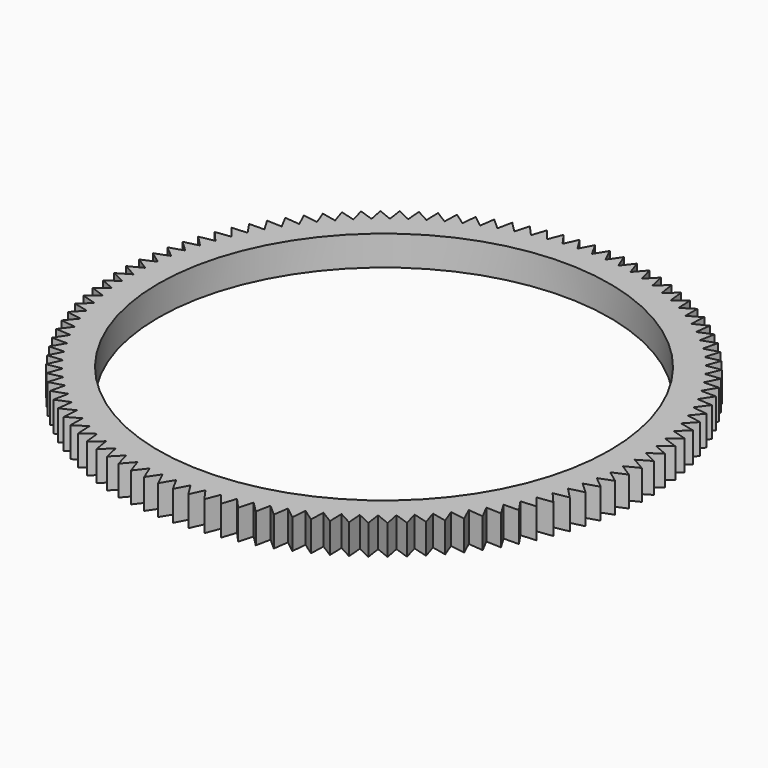
from build123d import *

# Parameters (mm, degrees)
F0_R     = 37.75
F1_DEPTH = 5


with BuildPart() as f1:
    # F0 (on Top) → F1 (new body)
    with BuildSketch(Plane.XY):
        with BuildLine():
            ThreePointArc((41.8418406427, -0.0778736447), (41.8418949929, -0.0389368392), (41.8419131096, 0))
            ThreePointArc((41.8419131096, 0), (41.8419099553, 0.016247102), (41.8419004922, 0.0324942016))
            ThreePointArc((41.8419004922, 0.0324942016), (41.8254914573, 1.1721591321), (41.7780466629, 2.3109542857))
            ThreePointArc((41.7780466629, 2.3109542857), (41.7749624862, 2.3660519757), (41.7718056457, 2.4211455503))
            ThreePointArc((41.7718056457, 2.4211455503), (41.6903612565, 3.5580150334), (41.5779813785, 4.6922443636))
            ThreePointArc((41.5779813785, 4.6922443636), (41.5717567702, 4.747076123), (41.5654598514, 4.8018996254))
            ThreePointArc((41.5654598514, 4.8018996254), (41.4192457627, 5.9322654293), (41.2422973609, 7.0582293156))
            ThreePointArc((41.2422973609, 7.0582293156), (41.2329526243, 7.1126162947), (41.2235361667, 7.166990902))
            ThreePointArc((41.2235361667, 7.166990902), (41.0130292983, 8.2871660083), (40.7720895416, 9.4011917907))
            ThreePointArc((40.7720895416, 9.4011917907), (40.7596551574, 9.4549565904), (40.7471498753, 9.508704944))
            ThreePointArc((40.7471498753, 9.508704944), (40.473036857, 10.6150355743), (40.1688916408, 11.7134895323))
            ThreePointArc((40.1688916408, 11.7134895323), (40.1534081673, 11.7664567829), (40.1378548505, 11.8194035669))
            ThreePointArc((40.1378548505, 11.8194035669), (39.8010297819, 12.9082811006), (39.4346711647, 13.9875803056))
            ThreePointArc((39.4346711647, 13.9875803056), (39.4161891058, 14.0395772391), (39.3976384858, 14.091549752))
            ThreePointArc((39.3976384858, 14.091549752), (38.9992000204, 15.159422497), (38.5718229878, 16.2160464994))
            ThreePointArc((38.5718229878, 16.2160464994), (38.5504026281, 16.2669035125), (38.5289152134, 16.3177322308))
            ThreePointArc((38.5289152134, 16.3177322308), (38.0701629745, 17.3611170082), (37.5831615416, 18.39161932))
            ThreePointArc((37.5831615416, 18.39161932), (37.5588727499, 18.4411705278), (37.5345186278, 18.4906896587))
            ThreePointArc((37.5345186278, 18.4906896587), (37.0169489699, 19.5061831642), (36.4719116342, 20.5072025011))
            ThreePointArc((36.4719116342, 20.5072025011), (36.4448336354, 20.5552862778), (36.4176922441, 20.6033343003))
            ThreePointArc((36.4176922441, 20.6033343003), (35.8429933719, 21.5876242051), (35.2416979318, 22.5558954502))
            ThreePointArc((35.2416979318, 22.5558954502), (35.2119190488, 22.6023549564), (35.1820789177, 22.6487751479))
            ThreePointArc((35.1820789177, 22.6487751479), (34.5521253795, 23.5986509029), (33.8965331358, 24.5310157565))
            ThreePointArc((33.8965331358, 24.5310157565), (33.8641505011, 24.5756994512), (33.8317089627, 24.6203403985))
            ThreePointArc((33.8317089627, 24.6203403985), (33.1485555358, 25.5327037065), (32.4408048942, 26.4261209884))
            ThreePointArc((32.4408048942, 26.4261209884), (32.4059241332, 26.4688831224), (32.370987005, 26.5115992162))
            ThreePointArc((32.370987005, 26.5115992162), (31.636861994, 27.3834741376), (30.8792614899, 28.2350297062))
            ThreePointArc((30.8792614899, 28.2350297062), (30.8419963764, 28.2757307985), (30.804677616, 28.3163827077))
            ThreePointArc((30.804677616, 28.3163827077), (30.0219755842, 29.1449253678), (29.216996353, 29.9518416259))
            ThreePointArc((29.216996353, 29.9518416259), (29.1774684381, 29.9903489179), (29.1378897715, 30.0288040444))
            ThreePointArc((29.1378897715, 30.0288040444), (28.3091637302, 30.8113119093), (27.4594314468, 31.5709568638))
            ThreePointArc((27.4594314468, 31.5709568638), (27.4177696623, 31.6071447527), (27.376060187, 31.6432776639))
            ThreePointArc((27.376060187, 31.6432776639), (26.5040132682, 32.3771983556), (25.6122995827, 33.0870942024))
            ThreePointArc((25.6122995827, 33.0870942024), (25.5686398207, 33.120844651), (25.5249355843, 33.1545374888))
            ThreePointArc((25.5249355843, 33.1545374888), (24.6124122238, 33.8374771104), (23.6816257209, 34.495308317))
            ThreePointArc((23.6816257209, 34.495308317), (23.6361103905, 34.5265112382), (23.5905539471, 34.5576541036))
            ThreePointArc((23.5905539471, 34.5576541036), (22.6405306065, 35.1873850482), (21.6737073184, 35.7910059058))
            ThreePointArc((21.6737073184, 35.7910059058), (21.626484881, 35.8195595222), (21.5792248263, 35.8480508336))
            ThreePointArc((21.5792248263, 35.8480508336), (20.5948002843, 36.4225190497), (19.5950937874, 36.9699606726))
            ThreePointArc((19.5950937874, 36.9699606726), (19.546318273, 36.9957718482), (19.4975087594, 37.0215186729))
            ThreePointArc((19.4975087594, 37.0215186729), (18.4818940042, 37.5388503646), (17.4525651335, 38.028327112))
            ThreePointArc((17.4525651335, 38.028327112), (17.4023956375, 38.0513116561), (17.3521958716, 38.0742300133))
            ThreePointArc((17.3521958716, 38.0742300133), (16.3087036273, 38.5327377521), (15.2531098396, 38.9626530526))
            ThreePointArc((15.2531098396, 38.9626530526), (15.2017100045, 38.9827359944), (15.1502837275, 39.0027511293))
            ThreePointArc((15.1502837275, 39.0027511293), (14.082317649, 39.4009393582), (13.0039020718, 39.7698909174))
            ThreePointArc((13.0039020718, 39.7698909174), (12.9514395533, 39.7870067506), (12.8989545069, 39.8040533778))
            ThreePointArc((12.8989545069, 39.8040533778), (11.8099980777, 40.1406232896), (10.7122782784, 40.4474076643))
            ThreePointArc((10.7122782784, 40.4474076643), (10.6589241982, 40.4615005606), (10.6055515778, 40.4755230776))
            ThreePointArc((10.6055515778, 40.4755230776), (9.4991567473, 40.7493768513), (8.3857132597, 40.9929933745))
            ThreePointArc((8.3857132597, 40.9929933745), (8.3316416478, 41.0040173657), (8.2775555438, 41.0149700341))
            ThreePointArc((8.2775555438, 41.0149700341), (7.157331142, 41.2252144154), (6.0317957875, 41.4048684608))
            ThreePointArc((6.0317957875, 41.4048684608), (5.9771830142, 41.412787589), (5.9225598441, 41.4206346833))
            ThreePointArc((5.9225598441, 41.4206346833), (4.7921598102, 41.5665838989), (3.658203851, 41.6816894722))
            ThreePointArc((3.658203851, 41.6816894722), (3.6032280519, 41.6864779069), (3.5482459853, 41.6911938316))
            ThreePointArc((3.5482459853, 41.6911938316), (2.4113574491, 41.7723718255), (1.272679614, 41.8225534763))
            ThreePointArc((1.272679614, 41.8225534763), (1.2175201087, 41.8241955985), (1.1623584855, 41.8257649712))
            ThreePointArc((1.1623584855, 41.8257649712), (0.0226897413, 41.8419069576), (-1.1169958394, 41.8270010038))
            ThreePointArc((-1.1169958394, 41.8270010038), (-1.1721591321, 41.8254914573), (-1.227320386, 41.8239091591))
            ThreePointArc((-1.227320386, 41.8239091591), (-2.3660519757, 41.7749624862), (-3.5030278845, 41.6950175478))
            ThreePointArc((-3.5030278845, 41.6950175478), (-3.5580150334, 41.6903612565), (-3.6129959935, 41.6856324484))
            ThreePointArc((-3.6129959935, 41.6856324484), (-4.747076123, 41.5717567702), (-5.8776337808, 41.4270336111))
            ThreePointArc((-5.8776337808, 41.4270336111), (-5.9322654293, 41.4192457627), (-5.9868867591, 41.4113858692))
            ThreePointArc((-5.9868867591, 41.4113858692), (-7.1126162947, 41.2329526243), (-8.2330680574, 41.0239233014))
            ThreePointArc((-8.2330680574, 41.0239233014), (-8.2871660083, 41.0130292983), (-8.3412495444, 41.0020639567))
            ThreePointArc((-8.3412495444, 41.0020639567), (-9.4549565904, 40.7596551574), (-10.5616477772, 40.4870014808))
            ThreePointArc((-10.5616477772, 40.4870014808), (-10.6150355743, 40.473036857), (-10.6684049075, 40.459001834))
            ThreePointArc((-10.6684049075, 40.459001834), (-11.7664567829, 40.1534081673), (-12.8557775972, 39.8180194767))
            ThreePointArc((-12.8557775972, 39.8180194767), (-12.9082811006, 39.8010297819), (-12.9607621512, 39.7839708568))
            ThreePointArc((-12.9607621512, 39.7839708568), (-14.0395772391, 39.4161891058), (-15.1079745429, 39.0191593693))
            ThreePointArc((-15.1079745429, 39.0191593693), (-15.159422497, 38.9992000204), (-15.2108440827, 38.9791728358))
            ThreePointArc((-15.2108440827, 38.9791728358), (-16.2669035125, 38.5504026281), (-17.3108924158, 38.0930268743))
            ThreePointArc((-17.3108924158, 38.0930268743), (-17.3611170082, 38.0701629745), (-17.4113114024, 38.047232855))
            ThreePointArc((-17.4113114024, 38.047232855), (-18.4411705278, 37.5588727499), (-19.4573457557, 37.0426428433))
            ThreePointArc((-19.4573457557, 37.0426428433), (-19.5061831642, 37.0169489699), (-19.5549866433, 36.9911907088))
            ThreePointArc((-19.5549866433, 36.9911907088), (-20.5552862778, 36.4448336354), (-21.540333278, 35.8714334108))
            ThreePointArc((-21.540333278, 35.8714334108), (-21.5876242051, 35.8429933719), (-21.6348775824, 35.8144909872))
            ThreePointArc((-21.6348775824, 35.8144909872), (-22.6023549564, 35.2119190488), (-23.5530607104, 34.5832188185))
            ThreePointArc((-23.5530607104, 34.5832188185), (-23.5986509029, 34.5521253795), (-23.6442000476, 34.5209718401))
            ThreePointArc((-23.6442000476, 34.5209718401), (-24.5756994512, 33.8641505011), (-25.4889629543, 33.1822009545))
            ThreePointArc((-25.4889629543, 33.1822009545), (-25.5327037065, 33.1485555358), (-25.5764000467, 33.1148524581))
            ThreePointArc((-25.5764000467, 33.1148524581), (-26.4688831224, 32.4059241332), (-27.341725499, 31.6729496481))
            ThreePointArc((-27.341725499, 31.6729496481), (-27.3834741376, 31.636861994), (-27.425175145, 31.6007193105))
            ThreePointArc((-27.425175145, 31.6007193105), (-28.2757307985, 30.8419963764), (-29.1053050182, 30.0603877632))
            ThreePointArc((-29.1053050182, 30.0603877632), (-29.1449253678, 30.0219755842), (-29.1844950224, 29.9835111847))
            ThreePointArc((-29.1844950224, 29.9835111847), (-29.9903489179, 29.1774684381), (-30.773949082, 28.3497751415))
            ThreePointArc((-30.773949082, 28.3497751415), (-30.8113119093, 28.3091637302), (-30.8486211431, 28.2685030775))
            ThreePointArc((-30.8486211431, 28.2685030775), (-31.6071447527, 27.4177696623), (-32.3422149203, 26.5466914459))
            ThreePointArc((-32.3422149203, 26.5466914459), (-32.3771983556, 26.5040132682), (-32.4121254735, 26.4612889891))
            ThreePointArc((-32.4121254735, 26.4612889891), (-33.120844651, 25.5686398207), (-33.804987176, 24.6570179606))
            ThreePointArc((-33.804987176, 24.6570179606), (-33.8374771104, 24.6124122238), (-33.8699081876, 24.5677636759))
            ThreePointArc((-33.8699081876, 24.5677636759), (-34.5265112382, 23.6361103905), (-35.1574945899, 22.6869184077))
            ThreePointArc((-35.1574945899, 22.6869184077), (-35.1873850482, 22.6405306065), (-35.2172143012, 22.5941034241))
            ThreePointArc((-35.2172143012, 22.5941034241), (-35.8195595222, 21.626484881), (-36.395325564, 20.6428188425))
            ThreePointArc((-36.395325564, 20.6428188425), (-36.4225190497, 20.5948002843), (-36.4496491816, 20.5467459032))
            ThreePointArc((-36.4496491816, 20.5467459032), (-36.9957718482, 19.546318273), (-37.514442551, 18.5313866929))
            ThreePointArc((-37.514442551, 18.5313866929), (-37.5388503646, 18.4818940042), (-37.5631928826, 18.4323691678))
            ThreePointArc((-37.5631928826, 18.4323691678), (-38.0513116561, 17.4023956375), (-38.5111952239, 16.3595090116))
            ThreePointArc((-38.5111952239, 16.3595090116), (-38.5327377521, 16.3087036273), (-38.554213256, 16.2578698755))
            ThreePointArc((-38.554213256, 16.2578698755), (-38.9827359944, 15.2017100045), (-39.3823323826, 14.1342700124))
            ThreePointArc((-39.3823323826, 14.1342700124), (-39.4009393582, 14.082317649), (-39.4194777993, 14.0303407908))
            ThreePointArc((-39.4194777993, 14.0303407908), (-39.7870067506, 12.9514395533), (-40.1250125587, 11.8629279622))
            ThreePointArc((-40.1250125587, 11.8629279622), (-40.1406232896, 11.8099980777), (-40.1561641995, 11.7570476507))
            ThreePointArc((-40.1561641995, 11.7570476507), (-40.4615005606, 10.6589241982), (-40.736813284, 9.5528915067))
            ThreePointArc((-40.736813284, 9.5528915067), (-40.7493768513, 9.4991567473), (-40.7618695386, 9.4454054649))
            ThreePointArc((-40.7618695386, 9.4454054649), (-41.0040173657, 8.3316416478), (-41.2157389916, 7.2116955047))
            ThreePointArc((-41.2157389916, 7.2116955047), (-41.2252144154, 7.157331142), (-41.2346181317, 7.1029543297))
            ThreePointArc((-41.2346181317, 7.1029543297), (-41.412787589, 5.9771830142), (-41.5602275253, 4.846976451))
            ThreePointArc((-41.5602275253, 4.846976451), (-41.5665838989, 4.7921598102), (-41.5728679712, 4.7373348338))
            ThreePointArc((-41.5728679712, 4.7373348338), (-41.6864779069, 3.6032280519), (-41.7691552353, 2.4664475675))
            ThreePointArc((-41.7691552353, 2.4664475675), (-41.7723718255, 2.4113574491), (-41.7755157563, 2.3562631364))
            ThreePointArc((-41.7755157563, 2.3562631364), (-41.8241955985, 1.2175201087), (-41.8418406427, 0.0778736447))
            ThreePointArc((-41.8418406427, 0.0778736447), (-41.8419069576, 0.0226897413), (-41.8419004922, -0.0324942016))
            ThreePointArc((-41.8419004922, -0.0324942016), (-41.8254914573, -1.1721591321), (-41.7780466629, -2.3109542857))
            ThreePointArc((-41.7780466629, -2.3109542857), (-41.7749624862, -2.3660519757), (-41.7718056457, -2.4211455503))
            ThreePointArc((-41.7718056457, -2.4211455503), (-41.6903612565, -3.5580150334), (-41.5779813785, -4.6922443636))
            ThreePointArc((-41.5779813785, -4.6922443636), (-41.5717567702, -4.747076123), (-41.5654598514, -4.8018996254))
            ThreePointArc((-41.5654598514, -4.8018996254), (-41.4192457627, -5.9322654293), (-41.2422973609, -7.0582293156))
            ThreePointArc((-41.2422973609, -7.0582293156), (-41.2329526243, -7.1126162947), (-41.2235361667, -7.166990902))
            ThreePointArc((-41.2235361667, -7.166990902), (-41.0130292983, -8.2871660083), (-40.7720895416, -9.4011917907))
            ThreePointArc((-40.7720895416, -9.4011917907), (-40.7596551574, -9.4549565904), (-40.7471498753, -9.508704944))
            ThreePointArc((-40.7471498753, -9.508704944), (-40.473036857, -10.6150355743), (-40.1688916408, -11.7134895323))
            ThreePointArc((-40.1688916408, -11.7134895323), (-40.1534081673, -11.7664567829), (-40.1378548505, -11.8194035669))
            ThreePointArc((-40.1378548505, -11.8194035669), (-39.8010297819, -12.9082811006), (-39.4346711647, -13.9875803056))
            ThreePointArc((-39.4346711647, -13.9875803056), (-39.4161891058, -14.0395772391), (-39.3976384858, -14.091549752))
            ThreePointArc((-39.3976384858, -14.091549752), (-38.9992000204, -15.159422497), (-38.5718229878, -16.2160464994))
            ThreePointArc((-38.5718229878, -16.2160464994), (-38.5504026281, -16.2669035125), (-38.5289152134, -16.3177322308))
            ThreePointArc((-38.5289152134, -16.3177322308), (-38.0701629745, -17.3611170082), (-37.5831615416, -18.39161932))
            ThreePointArc((-37.5831615416, -18.39161932), (-37.5588727499, -18.4411705278), (-37.5345186278, -18.4906896587))
            ThreePointArc((-37.5345186278, -18.4906896587), (-37.0169489699, -19.5061831642), (-36.4719116342, -20.5072025011))
            ThreePointArc((-36.4719116342, -20.5072025011), (-36.4448336354, -20.5552862778), (-36.4176922441, -20.6033343003))
            ThreePointArc((-36.4176922441, -20.6033343003), (-35.8429933719, -21.5876242051), (-35.2416979318, -22.5558954502))
            ThreePointArc((-35.2416979318, -22.5558954502), (-35.2119190488, -22.6023549564), (-35.1820789177, -22.6487751479))
            ThreePointArc((-35.1820789177, -22.6487751479), (-34.5521253795, -23.5986509029), (-33.8965331358, -24.5310157565))
            ThreePointArc((-33.8965331358, -24.5310157565), (-33.8641505011, -24.5756994512), (-33.8317089627, -24.6203403985))
            ThreePointArc((-33.8317089627, -24.6203403985), (-33.1485555358, -25.5327037065), (-32.4408048942, -26.4261209884))
            ThreePointArc((-32.4408048942, -26.4261209884), (-32.4059241332, -26.4688831224), (-32.370987005, -26.5115992162))
            ThreePointArc((-32.370987005, -26.5115992162), (-31.636861994, -27.3834741376), (-30.8792614899, -28.2350297062))
            ThreePointArc((-30.8792614899, -28.2350297062), (-30.8419963764, -28.2757307985), (-30.804677616, -28.3163827077))
            ThreePointArc((-30.804677616, -28.3163827077), (-30.0219755842, -29.1449253678), (-29.216996353, -29.9518416259))
            ThreePointArc((-29.216996353, -29.9518416259), (-29.1774684381, -29.9903489179), (-29.1378897715, -30.0288040444))
            ThreePointArc((-29.1378897715, -30.0288040444), (-28.3091637302, -30.8113119093), (-27.4594314468, -31.5709568638))
            ThreePointArc((-27.4594314468, -31.5709568638), (-27.4177696623, -31.6071447527), (-27.376060187, -31.6432776639))
            ThreePointArc((-27.376060187, -31.6432776639), (-26.5040132682, -32.3771983556), (-25.6122995827, -33.0870942024))
            ThreePointArc((-25.6122995827, -33.0870942024), (-25.5686398207, -33.120844651), (-25.5249355843, -33.1545374888))
            ThreePointArc((-25.5249355843, -33.1545374888), (-24.6124122238, -33.8374771104), (-23.6816257209, -34.495308317))
            ThreePointArc((-23.6816257209, -34.495308317), (-23.6361103905, -34.5265112382), (-23.5905539471, -34.5576541036))
            ThreePointArc((-23.5905539471, -34.5576541036), (-22.6405306065, -35.1873850482), (-21.6737073184, -35.7910059058))
            ThreePointArc((-21.6737073184, -35.7910059058), (-21.626484881, -35.8195595222), (-21.5792248263, -35.8480508336))
            ThreePointArc((-21.5792248263, -35.8480508336), (-20.5948002843, -36.4225190497), (-19.5950937874, -36.9699606726))
            ThreePointArc((-19.5950937874, -36.9699606726), (-19.546318273, -36.9957718482), (-19.4975087594, -37.0215186729))
            ThreePointArc((-19.4975087594, -37.0215186729), (-18.4818940042, -37.5388503646), (-17.4525651335, -38.028327112))
            ThreePointArc((-17.4525651335, -38.028327112), (-17.4023956375, -38.0513116561), (-17.3521958716, -38.0742300133))
            ThreePointArc((-17.3521958716, -38.0742300133), (-16.3087036273, -38.5327377521), (-15.2531098396, -38.9626530526))
            ThreePointArc((-15.2531098396, -38.9626530526), (-15.2017100045, -38.9827359944), (-15.1502837275, -39.0027511293))
            ThreePointArc((-15.1502837275, -39.0027511293), (-14.082317649, -39.4009393582), (-13.0039020718, -39.7698909174))
            ThreePointArc((-13.0039020718, -39.7698909174), (-12.9514395533, -39.7870067506), (-12.8989545069, -39.8040533778))
            ThreePointArc((-12.8989545069, -39.8040533778), (-11.8099980777, -40.1406232896), (-10.7122782784, -40.4474076643))
            ThreePointArc((-10.7122782784, -40.4474076643), (-10.6589241982, -40.4615005606), (-10.6055515778, -40.4755230776))
            ThreePointArc((-10.6055515778, -40.4755230776), (-9.4991567473, -40.7493768513), (-8.3857132597, -40.9929933745))
            ThreePointArc((-8.3857132597, -40.9929933745), (-8.3316416478, -41.0040173657), (-8.2775555438, -41.0149700341))
            ThreePointArc((-8.2775555438, -41.0149700341), (-7.157331142, -41.2252144154), (-6.0317957875, -41.4048684608))
            ThreePointArc((-6.0317957875, -41.4048684608), (-5.9771830142, -41.412787589), (-5.9225598441, -41.4206346833))
            ThreePointArc((-5.9225598441, -41.4206346833), (-4.7921598102, -41.5665838989), (-3.658203851, -41.6816894722))
            ThreePointArc((-3.658203851, -41.6816894722), (-3.6032280519, -41.6864779069), (-3.5482459853, -41.6911938316))
            ThreePointArc((-3.5482459853, -41.6911938316), (-2.4113574491, -41.7723718255), (-1.272679614, -41.8225534763))
            ThreePointArc((-1.272679614, -41.8225534763), (-1.2175201087, -41.8241955985), (-1.1623584855, -41.8257649712))
            ThreePointArc((-1.1623584855, -41.8257649712), (-0.0226897413, -41.8419069576), (1.1169958394, -41.8270010038))
            ThreePointArc((1.1169958394, -41.8270010038), (1.1721591321, -41.8254914573), (1.227320386, -41.8239091591))
            ThreePointArc((1.227320386, -41.8239091591), (2.3660519757, -41.7749624862), (3.5030278845, -41.6950175478))
            ThreePointArc((3.5030278845, -41.6950175478), (3.5580150334, -41.6903612565), (3.6129959935, -41.6856324484))
            ThreePointArc((3.6129959935, -41.6856324484), (4.747076123, -41.5717567702), (5.8776337808, -41.4270336111))
            ThreePointArc((5.8776337808, -41.4270336111), (5.9322654293, -41.4192457627), (5.9868867591, -41.4113858692))
            ThreePointArc((5.9868867591, -41.4113858692), (7.1126162947, -41.2329526243), (8.2330680574, -41.0239233014))
            ThreePointArc((8.2330680574, -41.0239233014), (8.2871660083, -41.0130292983), (8.3412495444, -41.0020639567))
            ThreePointArc((8.3412495444, -41.0020639567), (9.4549565904, -40.7596551574), (10.5616477772, -40.4870014808))
            ThreePointArc((10.5616477772, -40.4870014808), (10.6150355743, -40.473036857), (10.6684049075, -40.459001834))
            ThreePointArc((10.6684049075, -40.459001834), (11.7664567829, -40.1534081673), (12.8557775972, -39.8180194767))
            ThreePointArc((12.8557775972, -39.8180194767), (12.9082811006, -39.8010297819), (12.9607621512, -39.7839708568))
            ThreePointArc((12.9607621512, -39.7839708568), (14.0395772391, -39.4161891058), (15.1079745429, -39.0191593693))
            ThreePointArc((15.1079745429, -39.0191593693), (15.159422497, -38.9992000204), (15.2108440827, -38.9791728358))
            ThreePointArc((15.2108440827, -38.9791728358), (16.2669035125, -38.5504026281), (17.3108924158, -38.0930268743))
            ThreePointArc((17.3108924158, -38.0930268743), (17.3611170082, -38.0701629745), (17.4113114024, -38.047232855))
            ThreePointArc((17.4113114024, -38.047232855), (18.4411705278, -37.5588727499), (19.4573457557, -37.0426428433))
            ThreePointArc((19.4573457557, -37.0426428433), (19.5061831642, -37.0169489699), (19.5549866433, -36.9911907088))
            ThreePointArc((19.5549866433, -36.9911907088), (20.5552862778, -36.4448336354), (21.540333278, -35.8714334108))
            ThreePointArc((21.540333278, -35.8714334108), (21.5876242051, -35.8429933719), (21.6348775824, -35.8144909872))
            ThreePointArc((21.6348775824, -35.8144909872), (22.6023549564, -35.2119190488), (23.5530607104, -34.5832188185))
            ThreePointArc((23.5530607104, -34.5832188185), (23.5986509029, -34.5521253795), (23.6442000476, -34.5209718401))
            ThreePointArc((23.6442000476, -34.5209718401), (24.5756994512, -33.8641505011), (25.4889629543, -33.1822009545))
            ThreePointArc((25.4889629543, -33.1822009545), (25.5327037065, -33.1485555358), (25.5764000467, -33.1148524581))
            ThreePointArc((25.5764000467, -33.1148524581), (26.4688831224, -32.4059241332), (27.341725499, -31.6729496481))
            ThreePointArc((27.341725499, -31.6729496481), (27.3834741376, -31.636861994), (27.425175145, -31.6007193105))
            ThreePointArc((27.425175145, -31.6007193105), (28.2757307985, -30.8419963764), (29.1053050182, -30.0603877632))
            ThreePointArc((29.1053050182, -30.0603877632), (29.1449253678, -30.0219755842), (29.1844950224, -29.9835111847))
            ThreePointArc((29.1844950224, -29.9835111847), (29.9903489179, -29.1774684381), (30.773949082, -28.3497751415))
            ThreePointArc((30.773949082, -28.3497751415), (30.8113119093, -28.3091637302), (30.8486211431, -28.2685030775))
            ThreePointArc((30.8486211431, -28.2685030775), (31.6071447527, -27.4177696623), (32.3422149203, -26.5466914459))
            ThreePointArc((32.3422149203, -26.5466914459), (32.3771983556, -26.5040132682), (32.4121254735, -26.4612889891))
            ThreePointArc((32.4121254735, -26.4612889891), (33.120844651, -25.5686398207), (33.804987176, -24.6570179606))
            ThreePointArc((33.804987176, -24.6570179606), (33.8374771104, -24.6124122238), (33.8699081876, -24.5677636759))
            ThreePointArc((33.8699081876, -24.5677636759), (34.5265112382, -23.6361103905), (35.1574945899, -22.6869184077))
            ThreePointArc((35.1574945899, -22.6869184077), (35.1873850482, -22.6405306065), (35.2172143012, -22.5941034241))
            ThreePointArc((35.2172143012, -22.5941034241), (35.8195595222, -21.626484881), (36.395325564, -20.6428188425))
            ThreePointArc((36.395325564, -20.6428188425), (36.4225190497, -20.5948002843), (36.4496491816, -20.5467459032))
            ThreePointArc((36.4496491816, -20.5467459032), (36.9957718482, -19.546318273), (37.514442551, -18.5313866929))
            ThreePointArc((37.514442551, -18.5313866929), (37.5388503646, -18.4818940042), (37.5631928826, -18.4323691678))
            ThreePointArc((37.5631928826, -18.4323691678), (38.0513116561, -17.4023956375), (38.5111952239, -16.3595090116))
            ThreePointArc((38.5111952239, -16.3595090116), (38.5327377521, -16.3087036273), (38.554213256, -16.2578698755))
            ThreePointArc((38.554213256, -16.2578698755), (38.9827359944, -15.2017100045), (39.3823323826, -14.1342700124))
            ThreePointArc((39.3823323826, -14.1342700124), (39.4009393582, -14.082317649), (39.4194777993, -14.0303407908))
            ThreePointArc((39.4194777993, -14.0303407908), (39.7870067506, -12.9514395533), (40.1250125587, -11.8629279622))
            ThreePointArc((40.1250125587, -11.8629279622), (40.1406232896, -11.8099980777), (40.1561641995, -11.7570476507))
            ThreePointArc((40.1561641995, -11.7570476507), (40.4615005606, -10.6589241982), (40.736813284, -9.5528915067))
            ThreePointArc((40.736813284, -9.5528915067), (40.7493768513, -9.4991567473), (40.7618695386, -9.4454054649))
            ThreePointArc((40.7618695386, -9.4454054649), (41.0040173657, -8.3316416478), (41.2157389916, -7.2116955047))
            ThreePointArc((41.2157389916, -7.2116955047), (41.2252144154, -7.157331142), (41.2346181317, -7.1029543297))
            ThreePointArc((41.2346181317, -7.1029543297), (41.412787589, -5.9771830142), (41.5602275253, -4.846976451))
            ThreePointArc((41.5602275253, -4.846976451), (41.5665838989, -4.7921598102), (41.5728679712, -4.7373348338))
            ThreePointArc((41.5728679712, -4.7373348338), (41.6864779069, -3.6032280519), (41.7691552353, -2.4664475675))
            ThreePointArc((41.7691552353, -2.4664475675), (41.7723718255, -2.4113574491), (41.7755157563, -2.3562631364))
            ThreePointArc((41.7755157563, -2.3562631364), (41.8241955985, -1.2175201087), (41.8418406427, -0.0778736447))
        make_face()
        Circle(F0_R, mode=Mode.SUBTRACT)
        with BuildLine():
            ThreePointArc((38.5718229878, 16.2160464994), (38.9992000204, 15.159422497), (39.3976384858, 14.091549752))
            Line((39.3976384858, 14.091549752), (39.5059179026, 14.0726204482))
            Line((39.5059179026, 14.0726204482), (41.132787113, 16.0144523657))
            Line((41.132787113, 16.0144523657), (38.6380986891, 16.3050153419))
            Line((38.6380986891, 16.3050153419), (38.5718229878, 16.2160464994))
        make_face()
        with BuildLine():
            ThreePointArc((19.5950937874, 36.9699606726), (20.5948002843, 36.4225190497), (21.5792248263, 35.8480508336))
            Line((21.5792248263, 35.8480508336), (21.6750309134, 35.9019390912))
            Line((21.6750309134, 35.9019390912), (21.7052542773, 38.4350204504))
            Line((21.7052542773, 38.4350204504), (19.5900821802, 37.0807884999))
            Line((19.5900821802, 37.0807884999), (19.5950937874, 36.9699606726))
        make_face()
        with BuildLine():
            ThreePointArc((-39.3823323826, 14.1342700124), (-38.9827359944, 15.2017100045), (-38.554213256, 16.2578698755))
            Line((-38.554213256, 16.2578698755), (-38.6211876366, 16.3450316961))
            Line((-38.6211876366, 16.3450316961), (-41.132787113, 16.0144523657))
            Line((-41.132787113, 16.0144523657), (-39.4913189163, 14.1135369718))
            Line((-39.4913189163, 14.1135369718), (-39.3823323826, 14.1342700124))
        make_face()
        with BuildLine():
            ThreePointArc((-41.7691552353, 2.4664475675), (-41.6864779069, 3.6032280519), (-41.5728679712, 4.7373348338))
            Line((-41.5728679712, 4.7373348338), (-41.6616857413, 4.8020971248))
            Line((-41.6616857413, 4.8020971248), (-43.9784128316, 3.7773092378))
            Line((-43.9784128316, 3.7773092378), (-41.8678858761, 2.415849306))
            Line((-41.8678858761, 2.415849306), (-41.7691552353, 2.4664475675))
        make_face()
        with BuildLine():
            ThreePointArc((-30.773949082, 28.3497751415), (-29.9903489179, 29.1774684381), (-29.1844950224, 29.9835111847))
            Line((-29.1844950224, 29.9835111847), (-29.2122572173, 30.0898691236))
            Line((-29.2122572173, 30.0898691236), (-31.6544355533, 30.7630552784))
            Line((-31.6544355533, 30.7630552784), (-30.882409909, 28.373102647))
            Line((-30.882409909, 28.373102647), (-30.773949082, 28.3497751415))
        make_face()
        with BuildLine():
            ThreePointArc((-29.1053050182, 30.0603877632), (-28.2757307985, 30.8419963764), (-27.425175145, 31.6007193105))
            Line((-27.425175145, 31.6007193105), (-27.4468202144, 31.7084887013))
            Line((-27.4468202144, 31.7084887013), (-29.8465842143, 32.5199980166))
            Line((-29.8465842143, 32.5199980166), (-29.2122572173, 30.0898691236))
            Line((-29.2122572173, 30.0898691236), (-29.1053050182, 30.0603877632))
        make_face()
        with BuildLine():
            Line((41.6616857413, -4.8020971248), (41.5602275253, -4.846976451))
            ThreePointArc((41.5602275253, -4.846976451), (41.412787589, -5.9771830142), (41.2346181317, -7.1029543297))
            Line((41.2346181317, -7.1029543297), (41.3195938471, -7.172681501))
            Line((41.3195938471, -7.172681501), (43.6910465181, -6.2818241312))
            Line((43.6910465181, -6.2818241312), (41.6616857413, -4.8020971248))
        make_face()
        with BuildLine():
            Line((39.4913189163, -14.1135369718), (39.3823323826, -14.1342700124))
            ThreePointArc((39.3823323826, -14.1342700124), (38.9827359944, -15.2017100045), (38.554213256, -16.2578698755))
            Line((38.554213256, -16.2578698755), (38.6211876366, -16.3450316961))
            Line((38.6211876366, -16.3450316961), (41.132787113, -16.0144523657))
            Line((41.132787113, -16.0144523657), (39.4913189163, -14.1135369718))
        make_face()
        with BuildLine():
            Line((-37.6442500286, -18.4842266645), (-37.5831615416, -18.39161932))
            ThreePointArc((-37.5831615416, -18.39161932), (-38.0701629745, -17.3611170082), (-38.5289152134, -16.3177322308))
            Line((-38.5289152134, -16.3177322308), (-38.6380986891, -16.3050153419))
            Line((-38.6380986891, -16.3050153419), (-40.1514577699, -18.336556362))
            Line((-40.1514577699, -18.336556362), (-37.6442500286, -18.4842266645))
        make_face()
        with BuildLine():
            Line((-25.6262599804, -33.1971534174), (-25.6122995827, -33.0870942024))
            ThreePointArc((-25.6122995827, -33.0870942024), (-26.5040132682, -32.3771983556), (-27.376060187, -31.6432776639))
            Line((-27.376060187, -31.6432776639), (-27.4796522263, -31.6800396011))
            Line((-27.4796522263, -31.6800396011), (-27.9413795213, -34.1708672806))
            Line((-27.9413795213, -34.1708672806), (-25.6262599804, -33.1971534174))
        make_face()
        with BuildLine():
            Line((-27.4796522263, -31.6800396011), (-27.4594314468, -31.5709568638))
            ThreePointArc((-27.4594314468, -31.5709568638), (-28.3091637302, -30.8113119093), (-29.1378897715, -30.0288040444))
            Line((-29.1378897715, -30.0288040444), (-29.2434115582, -30.0595920804))
            Line((-29.2434115582, -30.0595920804), (-29.8465842143, -32.5199980166))
            Line((-29.8465842143, -32.5199980166), (-27.4796522263, -31.6800396011))
        make_face()
        with BuildLine():
            Line((-19.5900821802, -37.0807884999), (-19.5950937874, -36.9699606726))
            ThreePointArc((-19.5950937874, -36.9699606726), (-20.5948002843, -36.4225190497), (-21.5792248263, -35.8480508336))
            Line((-21.5792248263, -35.8480508336), (-21.6750309134, -35.9019390912))
            Line((-21.6750309134, -35.9019390912), (-21.7052542773, -38.4350204504))
            Line((-21.7052542773, -38.4350204504), (-19.5900821802, -37.0807884999))
        make_face()
        with BuildLine():
            Line((12.9387485344, -39.8916655702), (12.8557775972, -39.8180194767))
            ThreePointArc((12.8557775972, -39.8180194767), (11.7664567829, -40.1534081673), (10.6684049075, -40.459001834))
            Line((10.6684049075, -40.459001834), (10.6402790295, -40.5652641774))
            Line((10.6402790295, -40.5652641774), (12.4357684384, -42.3523378765))
            Line((12.4357684384, -42.3523378765), (12.9387485344, -39.8916655702))
        make_face()
        with BuildLine():
            Line((40.2326377221, -11.8360068234), (40.1250125587, -11.8629279622))
            ThreePointArc((40.1250125587, -11.8629279622), (39.7870067506, -12.9514395533), (39.4194777993, -14.0303407908))
            Line((39.4194777993, -14.0303407908), (39.4913189163, -14.1135369718))
            Line((39.4913189163, -14.1135369718), (41.9799498542, -13.6401125545))
            Line((41.9799498542, -13.6401125545), (40.2326377221, -11.8360068234))
        make_face()
        with BuildLine():
            Line((37.6250820702, -18.5232123244), (37.514442551, -18.5313866929))
            ThreePointArc((37.514442551, -18.5313866929), (36.9957718482, -19.546318273), (36.4496491816, -20.5467459032))
            Line((36.4496491816, -20.5467459032), (36.5062513066, -20.6409740841))
            Line((36.5062513066, -20.6409740841), (39.039162717, -20.5988503227))
            Line((39.039162717, -20.5988503227), (37.6250820702, -18.5232123244))
        make_face()
        with BuildLine():
            Line((33.9154001618, -24.6678298086), (33.804987176, -24.6570179606))
            ThreePointArc((33.804987176, -24.6570179606), (33.120844651, -25.5686398207), (32.4121254735, -26.4612889891))
            Line((32.4121254735, -26.4612889891), (32.4518305985, -26.563789007))
            Line((32.4518305985, -26.563789007), (34.9548276087, -26.9541998046))
            Line((34.9548276087, -26.9541998046), (33.9154001618, -24.6678298086))
        make_face()
        with BuildLine():
            Line((32.4518305985, -26.563789007), (32.3422149203, -26.5466914459))
            ThreePointArc((32.3422149203, -26.5466914459), (31.6071447527, -27.4177696623), (30.8486211431, -28.2685030775))
            Line((30.8486211431, -28.2685030775), (30.882409909, -28.373102647))
            Line((30.882409909, -28.373102647), (33.359036703, -28.9057698481))
            Line((33.359036703, -28.9057698481), (32.4518305985, -26.563789007))
        make_face()
        with BuildLine():
            Line((30.882409909, -28.373102647), (30.773949082, -28.3497751415))
            ThreePointArc((30.773949082, -28.3497751415), (29.9903489179, -29.1774684381), (29.1844950224, -29.9835111847))
            Line((29.1844950224, -29.9835111847), (29.2122572173, -30.0898691236))
            Line((29.2122572173, -30.0898691236), (31.6544355533, -30.7630552784))
            Line((31.6544355533, -30.7630552784), (30.882409909, -28.373102647))
        make_face()
        with BuildLine():
            Line((29.2122572173, -30.0898691236), (29.1053050182, -30.0603877632))
            ThreePointArc((29.1053050182, -30.0603877632), (28.2757307985, -30.8419963764), (27.425175145, -31.6007193105))
            Line((27.425175145, -31.6007193105), (27.4468202144, -31.7084887013))
            Line((27.4468202144, -31.7084887013), (29.8465842143, -32.5199980166))
            Line((29.8465842143, -32.5199980166), (29.2122572173, -30.0898691236))
        make_face()
        with BuildLine():
            Line((27.4468202144, -31.7084887013), (27.341725499, -31.6729496481))
            ThreePointArc((27.341725499, -31.6729496481), (26.4688831224, -32.4059241332), (25.5764000467, -33.1148524581))
            Line((25.5764000467, -33.1148524581), (25.5918573889, -33.2236817796))
            Line((25.5918573889, -33.2236817796), (27.9413795213, -34.1708672806))
            Line((27.9413795213, -34.1708672806), (27.4468202144, -31.7084887013))
        make_face()
        with BuildLine():
            Line((25.5918573889, -33.2236817796), (25.4889629543, -33.1822009545))
            ThreePointArc((25.4889629543, -33.1822009545), (24.5756994512, -33.8641505011), (23.6442000476, -34.5209718401))
            Line((23.6442000476, -34.5209718401), (23.6534192439, -34.6305061135))
            Line((23.6534192439, -34.6305061135), (25.9450358559, -35.7102782781))
            Line((25.9450358559, -35.7102782781), (25.5918573889, -33.2236817796))
        make_face()
        with BuildLine():
            Line((23.6534192439, -34.6305061135), (23.5530607104, -34.5832188185))
            ThreePointArc((23.5530607104, -34.5832188185), (22.6023549564, -35.2119190488), (21.6348775824, -35.8144909872))
            Line((21.6348775824, -35.8144909872), (21.6378285617, -35.9243729345))
            Line((21.6378285617, -35.9243729345), (23.8640648763, -37.1332097702))
            Line((23.8640648763, -37.1332097702), (23.6534192439, -34.6305061135))
        make_face()
        with BuildLine():
            Line((21.6378285617, -35.9243729345), (21.540333278, -35.8714334108))
            ThreePointArc((21.540333278, -35.8714334108), (20.5552862778, -36.4448336354), (19.5549866433, -36.9911907088))
            Line((19.5549866433, -36.9911907088), (19.5516597802, -37.101061918))
            Line((19.5516597802, -37.101061918), (21.7052542773, -38.4350204504))
            Line((21.7052542773, -38.4350204504), (21.6378285617, -35.9243729345))
        make_face()
        with BuildLine():
            Line((19.5516597802, -37.101061918), (19.4573457557, -37.0426428433))
            ThreePointArc((19.4573457557, -37.0426428433), (18.4411705278, -37.5588727499), (17.4113114024, -38.047232855))
            Line((17.4113114024, -38.047232855), (17.4017175484, -38.156734949))
            Line((17.4017175484, -38.156734949), (19.4756456503, -39.6114640826))
            Line((19.4756456503, -39.6114640826), (19.5516597802, -37.101061918))
        make_face()
        with BuildLine():
            Line((17.4017175484, -38.156734949), (17.3108924158, -38.0930268743))
            ThreePointArc((17.3108924158, -38.0930268743), (16.2669035125, -38.5504026281), (15.2108440827, -38.9791728358))
            Line((15.2108440827, -38.9791728358), (15.1950145309, -39.0879486416))
            Line((15.1950145309, -39.0879486416), (17.1825115153, -40.6587033523))
            Line((17.1825115153, -40.6587033523), (17.4017175484, -38.156734949))
        make_face()
        with BuildLine():
            ThreePointArc((36.4719116342, 20.5072025011), (37.0169489699, 19.5061831642), (37.5345186278, 18.4906896587))
            Line((37.5345186278, 18.4906896587), (37.6442500286, 18.4842266645))
            Line((37.6442500286, 18.4842266645), (39.039162717, 20.5988503227))
            Line((39.039162717, 20.5988503227), (36.5276136491, 20.6031462818))
            Line((36.5276136491, 20.6031462818), (36.4719116342, 20.5072025011))
        make_face()
        with BuildLine():
            Line((41.8678858761, -2.415849306), (41.7691552353, -2.4664475675))
            ThreePointArc((41.7691552353, -2.4664475675), (41.6864779069, -3.6032280519), (41.5728679712, -4.7373348338))
            Line((41.5728679712, -4.7373348338), (41.6616857413, -4.8020971248))
            Line((41.6616857413, -4.8020971248), (43.9784128316, -3.7773092378))
            Line((43.9784128316, -3.7773092378), (41.8678858761, -2.415849306))
        make_face()
        with BuildLine():
            ThreePointArc((35.2416979318, 22.5558954502), (35.8429933719, 21.5876242051), (36.4176922441, 20.6033343003))
            Line((36.4176922441, 20.6033343003), (36.5276136491, 20.6031462818))
            Line((36.5276136491, 20.6031462818), (37.7995300297, 22.7939551152))
            Line((37.7995300297, 22.7939551152), (35.2918317861, 22.6548627183))
            Line((35.2918317861, 22.6548627183), (35.2416979318, 22.5558954502))
        make_face()
        with BuildLine():
            Line((41.9375216695, -0.0217214888), (41.8418406427, -0.0778736447))
            ThreePointArc((41.8418406427, -0.0778736447), (41.8241955985, -1.2175201087), (41.7755157563, -2.3562631364))
            Line((41.7755157563, -2.3562631364), (41.8678858761, -2.415849306))
            Line((41.8678858761, -2.415849306), (44.1223307034, -1.2604735469))
            Line((44.1223307034, -1.2604735469), (41.9375216695, -0.0217214888))
        make_face()
        with BuildLine():
            ThreePointArc((33.8965331358, 24.5310157565), (34.5521253795, 23.5986509029), (35.1820789177, 22.6487751479))
            Line((35.1820789177, 22.6487751479), (35.2918317861, 22.6548627183))
            Line((35.2918317861, 22.6548627183), (36.4366031322, 24.9147107639))
            Line((36.4366031322, 24.9147107639), (33.9409353034, 24.6326837015))
            Line((33.9409353034, 24.6326837015), (33.8965331358, 24.5310157565))
        make_face()
        with BuildLine():
            ThreePointArc((32.4408048942, 26.4261209884), (33.1485555358, 25.5327037065), (33.8317089627, 24.6203403985))
            Line((33.8317089627, 24.6203403985), (33.9409353034, 24.6326837015))
            Line((33.9409353034, 24.6326837015), (34.9548276087, 26.9541998046))
            Line((34.9548276087, 26.9541998046), (32.4793305444, 26.5301579904))
            Line((32.4793305444, 26.5301579904), (32.4408048942, 26.4261209884))
        make_face()
        with BuildLine():
            ThreePointArc((30.8792614899, 28.2350297062), (31.636861994, 27.3834741376), (32.370987005, 26.5115992162))
            Line((32.370987005, 26.5115992162), (32.4793305444, 26.5301579904))
            Line((32.4793305444, 26.5301579904), (33.359036703, 28.9057698481))
            Line((33.359036703, 28.9057698481), (30.91178496, 28.3410964182))
            Line((30.91178496, 28.3410964182), (30.8792614899, 28.2350297062))
        make_face()
        with BuildLine():
            ThreePointArc((29.216996353, 29.9518416259), (30.0219755842, 29.1449253678), (30.804677616, 28.3163827077))
            Line((30.804677616, 28.3163827077), (30.91178496, 28.3410964182))
            Line((30.91178496, 28.3410964182), (31.6544355533, 30.7630552784))
            Line((31.6544355533, 30.7630552784), (29.2434115582, 30.0595920804))
            Line((29.2434115582, 30.0595920804), (29.216996353, 29.9518416259))
        make_face()
        with BuildLine():
            ThreePointArc((27.4594314468, 31.5709568638), (28.3091637302, 30.8113119093), (29.1378897715, 30.0288040444))
            Line((29.1378897715, 30.0288040444), (29.2434115582, 30.0595920804))
            Line((29.2434115582, 30.0595920804), (29.8465842143, 32.5199980166))
            Line((29.8465842143, 32.5199980166), (27.4796522263, 31.6800396011))
            Line((27.4796522263, 31.6800396011), (27.4594314468, 31.5709568638))
        make_face()
        with BuildLine():
            ThreePointArc((25.6122995827, 33.0870942024), (26.5040132682, 32.3771983556), (27.376060187, 31.6432776639))
            Line((27.376060187, 31.6432776639), (27.4796522263, 31.6800396011))
            Line((27.4796522263, 31.6800396011), (27.9413795213, 34.1708672806))
            Line((27.9413795213, 34.1708672806), (25.6262599804, 33.1971534174))
            Line((25.6262599804, 33.1971534174), (25.6122995827, 33.0870942024))
        make_face()
        with BuildLine():
            ThreePointArc((23.6816257209, 34.495308317), (24.6124122238, 33.8374771104), (25.5249355843, 33.1545374888))
            Line((25.5249355843, 33.1545374888), (25.6262599804, 33.1971534174))
            Line((25.6262599804, 33.1971534174), (25.9450358559, 35.7102782781))
            Line((25.9450358559, 35.7102782781), (23.689280201, 34.6059850194))
            Line((23.689280201, 34.6059850194), (23.6816257209, 34.495308317))
        make_face()
        with BuildLine():
            ThreePointArc((21.6737073184, 35.7910059058), (22.6405306065, 35.1873850482), (23.5905539471, 34.5576541036))
            Line((23.5905539471, 34.5576541036), (23.689280201, 34.6059850194))
            Line((23.689280201, 34.6059850194), (23.8640648763, 37.1332097702))
            Line((23.8640648763, 37.1332097702), (21.6750309134, 35.9019390912))
            Line((21.6750309134, 35.9019390912), (21.6737073184, 35.7910059058))
        make_face()
        with BuildLine():
            ThreePointArc((21.5792248263, 35.8480508336), (21.626484881, 35.8195595222), (21.6737073184, 35.7910059058))
            Line((21.6737073184, 35.7910059058), (21.6750309134, 35.9019390912))
            Line((21.6750309134, 35.9019390912), (21.5792248263, 35.8480508336))
        make_face()
        with BuildLine():
            ThreePointArc((17.4525651335, 38.028327112), (18.4818940042, 37.5388503646), (19.4975087594, 37.0215186729))
            Line((19.4975087594, 37.0215186729), (19.5900821802, 37.0807884999))
            Line((19.5900821802, 37.0807884999), (19.4756456503, 39.6114640826))
            Line((19.4756456503, 39.6114640826), (17.4412346708, 38.1386880839))
            Line((17.4412346708, 38.1386880839), (17.4525651335, 38.028327112))
        make_face()
        with BuildLine():
            ThreePointArc((15.2531098396, 38.9626530526), (16.3087036273, 38.5327377521), (17.3521958716, 38.0742300133))
            Line((17.3521958716, 38.0742300133), (17.4412346708, 38.1386880839))
            Line((17.4412346708, 38.1386880839), (17.1825115153, 40.6587033523))
            Line((17.1825115153, 40.6587033523), (15.2354974791, 39.0721871946))
            Line((15.2354974791, 39.0721871946), (15.2531098396, 38.9626530526))
        make_face()
        with BuildLine():
            ThreePointArc((13.0039020718, 39.7698909174), (14.082317649, 39.4009393582), (15.1502837275, 39.0027511293))
            Line((15.1502837275, 39.0027511293), (15.2354974791, 39.0721871946))
            Line((15.2354974791, 39.0721871946), (14.8333315991, 41.5733223827))
            Line((14.8333315991, 41.5733223827), (12.9800652613, 39.8782409519))
            Line((12.9800652613, 39.8782409519), (13.0039020718, 39.7698909174))
        make_face()
        with BuildLine():
            ThreePointArc((10.7122782784, 40.4474076643), (11.8099980777, 40.1406232896), (12.8989545069, 39.8040533778))
            Line((12.8989545069, 39.8040533778), (12.9800652613, 39.8782409519))
            Line((12.9800652613, 39.8782409519), (12.4357684384, 42.3523378765))
            Line((12.4357684384, 42.3523378765), (10.6822947686, 40.554220176))
            Line((10.6822947686, 40.554220176), (10.7122782784, 40.4474076643))
        make_face()
        with BuildLine():
            ThreePointArc((8.3857132597, 40.9929933745), (9.4991567473, 40.7493768513), (10.6055515778, 40.4755230776))
            Line((10.6055515778, 40.4755230776), (10.6822947686, 40.554220176))
            Line((10.6822947686, 40.554220176), (9.9976423859, 42.9932088473))
            Line((9.9976423859, 42.9932088473), (8.3496808507, 41.0979199631))
            Line((8.3496808507, 41.0979199631), (8.3857132597, 40.9929933745))
        make_face()
        with BuildLine():
            ThreePointArc((6.0317957875, 41.4048684608), (7.157331142, 41.2252144154), (8.2775555438, 41.0149700341))
            Line((8.2775555438, 41.0149700341), (8.3496808507, 41.0979199631))
            Line((8.3496808507, 41.0979199631), (7.5269061019, 43.493844907))
            Line((7.5269061019, 43.493844907), (5.9898320093, 41.5075668777))
            Line((5.9898320093, 41.5075668777), (6.0317957875, 41.4048684608))
        make_face()
        with BuildLine():
            ThreePointArc((3.658203851, 41.6816894722), (4.7921598102, 41.5665838989), (5.9225598441, 41.4206346833))
            Line((5.9225598441, 41.4206346833), (5.9898320093, 41.5075668777))
            Line((5.9898320093, 41.5075668777), (5.0316186147, 43.8526130849))
            Line((5.0316186147, 43.8526130849), (3.610445581, 41.7818247365))
            Line((3.610445581, 41.7818247365), (3.658203851, 41.6816894722))
        make_face()
        with BuildLine():
            ThreePointArc((1.272679614, 41.8225534763), (2.4113574491, 41.7723718255), (3.5482459853, 41.6911938316))
            Line((3.5482459853, 41.6911938316), (3.610445581, 41.7818247365))
            Line((3.610445581, 41.7818247365), (2.5199190334, 44.0683431539))
            Line((2.5199190334, 44.0683431539), (1.2192826296, 41.9197989675))
            Line((1.2192826296, 41.9197989675), (1.272679614, 41.8225534763))
        make_face()
        with BuildLine():
            ThreePointArc((-1.1169958394, 41.8270010038), (0.0226897413, 41.8419069576), (1.1623584855, 41.8257649712))
            Line((1.1623584855, 41.8257649712), (1.2192826296, 41.9197989675))
            Line((1.2192826296, 41.9197989675), (0, 44.1403314471))
            Line((0, 44.1403314471), (-1.1758573683, 41.9210395273))
            Line((-1.1758573683, 41.9210395273), (-1.1169958394, 41.8270010038))
        make_face()
        with BuildLine():
            ThreePointArc((-3.5030278845, 41.6950175478), (-2.3660519757, 41.7749624862), (-1.227320386, 41.8239091591))
            Line((-1.227320386, 41.8239091591), (-1.1758573683, 41.9210395273))
            Line((-1.1758573683, 41.9210395273), (-2.5199190334, 44.0683431539))
            Line((-2.5199190334, 44.0683431539), (-3.5671619639, 41.7855423697))
            Line((-3.5671619639, 41.7855423697), (-3.5030278845, 41.6950175478))
        make_face()
        with BuildLine():
            ThreePointArc((-5.8776337808, 41.4270336111), (-4.747076123, 41.5717567702), (-3.6129959935, 41.6856324484))
            Line((-3.6129959935, 41.6856324484), (-3.5671619639, 41.7855423697))
            Line((-3.5671619639, 41.7855423697), (-5.0316186147, 43.8526130849))
            Line((-5.0316186147, 43.8526130849), (-5.9468312186, 41.513749458))
            Line((-5.9468312186, 41.513749458), (-5.8776337808, 41.4270336111))
        make_face()
        with BuildLine():
            ThreePointArc((-8.2330680574, 41.0239233014), (-7.1126162947, 41.2329526243), (-5.9868867591, 41.4113858692))
            Line((-5.9868867591, 41.4113858692), (-5.9468312186, 41.513749458))
            Line((-5.9468312186, 41.513749458), (-7.5269061019, 43.493844907))
            Line((-7.5269061019, 43.493844907), (-8.3071031459, 41.1065473243))
            Line((-8.3071031459, 41.1065473243), (-8.2330680574, 41.0239233014))
        make_face()
        with BuildLine():
            ThreePointArc((-10.5616477772, 40.4870014808), (-9.4549565904, 40.7596551574), (-8.3412495444, 41.0020639567))
            Line((-8.3412495444, 41.0020639567), (-8.3071031459, 41.1065473243))
            Line((-8.3071031459, 41.1065473243), (-9.9976423859, 42.9932088473))
            Line((-9.9976423859, 42.9932088473), (-10.6402790295, 40.5652641774))
            Line((-10.6402790295, 40.5652641774), (-10.5616477772, 40.4870014808))
        make_face()
        with BuildLine():
            ThreePointArc((-12.8557775972, 39.8180194767), (-11.7664567829, 40.1534081673), (-10.6684049075, 40.459001834))
            Line((-10.6684049075, 40.459001834), (-10.6402790295, 40.5652641774))
            Line((-10.6402790295, 40.5652641774), (-12.4357684384, 42.3523378765))
            Line((-12.4357684384, 42.3523378765), (-12.9387485344, 39.8916655702))
            Line((-12.9387485344, 39.8916655702), (-12.8557775972, 39.8180194767))
        make_face()
        with BuildLine():
            ThreePointArc((-36.395325564, 20.6428188425), (-35.8195595222, 21.626484881), (-35.2172143012, 22.5941034241))
            Line((-35.2172143012, 22.5941034241), (-35.2683447392, 22.6914092767))
            Line((-35.2683447392, 22.6914092767), (-37.7995300297, 22.7939551152))
            Line((-37.7995300297, 22.7939551152), (-36.5062513066, 20.6409740841))
            Line((-36.5062513066, 20.6409740841), (-36.395325564, 20.6428188425))
        make_face()
        with BuildLine():
            ThreePointArc((-37.514442551, 18.5313866929), (-36.9957718482, 19.546318273), (-36.4496491816, 20.5467459032))
            Line((-36.4496491816, 20.5467459032), (-36.5062513066, 20.6409740841))
            Line((-36.5062513066, 20.6409740841), (-39.039162717, 20.5988503227))
            Line((-39.039162717, 20.5988503227), (-37.6250820702, 18.5232123244))
            Line((-37.6250820702, 18.5232123244), (-37.514442551, 18.5313866929))
        make_face()
        with BuildLine():
            ThreePointArc((-38.5111952239, 16.3595090116), (-38.0513116561, 17.4023956375), (-37.5631928826, 18.4323691678))
            Line((-37.5631928826, 18.4323691678), (-37.6250820702, 18.5232123244))
            Line((-37.6250820702, 18.5232123244), (-40.1514577699, 18.336556362))
            Line((-40.1514577699, 18.336556362), (-38.6211876366, 16.3450316961))
            Line((-38.6211876366, 16.3450316961), (-38.5111952239, 16.3595090116))
        make_face()
        with BuildLine():
            ThreePointArc((-38.554213256, 16.2578698755), (-38.5327377521, 16.3087036273), (-38.5111952239, 16.3595090116))
            Line((-38.5111952239, 16.3595090116), (-38.6211876366, 16.3450316961))
            Line((-38.6211876366, 16.3450316961), (-38.554213256, 16.2578698755))
        make_face()
        with BuildLine():
            ThreePointArc((-40.1250125587, 11.8629279622), (-39.7870067506, 12.9514395533), (-39.4194777993, 14.0303407908))
            Line((-39.4194777993, 14.0303407908), (-39.4913189163, 14.1135369718))
            Line((-39.4913189163, 14.1135369718), (-41.9799498542, 13.6401125545))
            Line((-41.9799498542, 13.6401125545), (-40.2326377221, 11.8360068234))
            Line((-40.2326377221, 11.8360068234), (-40.1250125587, 11.8629279622))
        make_face()
        with BuildLine():
            ThreePointArc((-40.736813284, 9.5528915067), (-40.4615005606, 10.6589241982), (-40.1561641995, 11.7570476507))
            Line((-40.1561641995, 11.7570476507), (-40.2326377221, 11.8360068234))
            Line((-40.2326377221, 11.8360068234), (-42.6901827246, 11.2212815312))
            Line((-42.6901827246, 11.2212815312), (-40.8427260261, 9.5198700809))
            Line((-40.8427260261, 9.5198700809), (-40.736813284, 9.5528915067))
        make_face()
        with BuildLine():
            ThreePointArc((-41.8418406427, 0.0778736447), (-41.8241955985, 1.2175201087), (-41.7755157563, 2.3562631364))
            Line((-41.7755157563, 2.3562631364), (-41.8678858761, 2.415849306))
            Line((-41.8678858761, 2.415849306), (-44.1223307034, 1.2604735469))
            Line((-44.1223307034, 1.2604735469), (-41.9375216695, 0.0217214888))
            Line((-41.9375216695, 0.0217214888), (-41.8418406427, 0.0778736447))
        make_face()
        with BuildLine():
            Line((-41.870365984, -2.3724771793), (-41.7780466629, -2.3109542857))
            ThreePointArc((-41.7780466629, -2.3109542857), (-41.8254914573, -1.1721591321), (-41.8419004922, -0.0324942016))
            Line((-41.8419004922, -0.0324942016), (-41.9375216695, 0.0217214888))
            Line((-41.9375216695, 0.0217214888), (-44.1223307034, -1.2604735469))
            Line((-44.1223307034, -1.2604735469), (-41.870365984, -2.3724771793))
        make_face()
        with BuildLine():
            ThreePointArc((-41.5602275253, 4.846976451), (-41.412787589, 5.9771830142), (-41.2346181317, 7.1029543297))
            Line((-41.2346181317, 7.1029543297), (-41.3195938471, 7.172681501))
            Line((-41.3195938471, 7.172681501), (-43.6910465181, 6.2818241312))
            Line((-43.6910465181, 6.2818241312), (-41.6616857413, 4.8020971248))
            Line((-41.6616857413, 4.8020971248), (-41.5602275253, 4.846976451))
        make_face()
        with BuildLine():
            ThreePointArc((-41.2157389916, 7.2116955047), (-41.0040173657, 8.3316416478), (-40.7618695386, 9.4454054649))
            Line((-40.7618695386, 9.4454054649), (-40.8427260261, 9.5198700809))
            Line((-40.8427260261, 9.5198700809), (-43.2611690922, 8.76584902))
            Line((-43.2611690922, 8.76584902), (-41.3195938471, 7.172681501))
            Line((-41.3195938471, 7.172681501), (-41.2157389916, 7.2116955047))
        make_face()
        with BuildLine():
            ThreePointArc((-35.1574945899, 22.6869184077), (-34.5265112382, 23.6361103905), (-33.8699081876, 24.5677636759))
            Line((-33.8699081876, 24.5677636759), (-33.9154001618, 24.6678298086))
            Line((-33.9154001618, 24.6678298086), (-36.4366031322, 24.9147107639))
            Line((-36.4366031322, 24.9147107639), (-35.2683447392, 22.6914092767))
            Line((-35.2683447392, 22.6914092767), (-35.1574945899, 22.6869184077))
        make_face()
        with BuildLine():
            ThreePointArc((-33.804987176, 24.6570179606), (-33.120844651, 25.5686398207), (-32.4121254735, 26.4612889891))
            Line((-32.4121254735, 26.4612889891), (-32.4518305985, 26.563789007))
            Line((-32.4518305985, 26.563789007), (-34.9548276087, 26.9541998046))
            Line((-34.9548276087, 26.9541998046), (-33.9154001618, 24.6678298086))
            Line((-33.9154001618, 24.6678298086), (-33.804987176, 24.6570179606))
        make_face()
        with BuildLine():
            ThreePointArc((-32.3422149203, 26.5466914459), (-31.6071447527, 27.4177696623), (-30.8486211431, 28.2685030775))
            Line((-30.8486211431, 28.2685030775), (-30.882409909, 28.373102647))
            Line((-30.882409909, 28.373102647), (-33.359036703, 28.9057698481))
            Line((-33.359036703, 28.9057698481), (-32.4518305985, 26.563789007))
            Line((-32.4518305985, 26.563789007), (-32.3422149203, 26.5466914459))
        make_face()
        with BuildLine():
            ThreePointArc((-29.1844950224, 29.9835111847), (-29.1449253678, 30.0219755842), (-29.1053050182, 30.0603877632))
            Line((-29.1053050182, 30.0603877632), (-29.2122572173, 30.0898691236))
            Line((-29.2122572173, 30.0898691236), (-29.1844950224, 29.9835111847))
        make_face()
        with BuildLine():
            ThreePointArc((-27.341725499, 31.6729496481), (-26.4688831224, 32.4059241332), (-25.5764000467, 33.1148524581))
            Line((-25.5764000467, 33.1148524581), (-25.5918573889, 33.2236817796))
            Line((-25.5918573889, 33.2236817796), (-27.9413795213, 34.1708672806))
            Line((-27.9413795213, 34.1708672806), (-27.4468202144, 31.7084887013))
            Line((-27.4468202144, 31.7084887013), (-27.341725499, 31.6729496481))
        make_face()
        with BuildLine():
            ThreePointArc((-25.4889629543, 33.1822009545), (-24.5756994512, 33.8641505011), (-23.6442000476, 34.5209718401))
            Line((-23.6442000476, 34.5209718401), (-23.6534192439, 34.6305061135))
            Line((-23.6534192439, 34.6305061135), (-25.9450358559, 35.7102782781))
            Line((-25.9450358559, 35.7102782781), (-25.5918573889, 33.2236817796))
            Line((-25.5918573889, 33.2236817796), (-25.4889629543, 33.1822009545))
        make_face()
        with BuildLine():
            ThreePointArc((-23.5530607104, 34.5832188185), (-22.6023549564, 35.2119190488), (-21.6348775824, 35.8144909872))
            Line((-21.6348775824, 35.8144909872), (-21.6378285617, 35.9243729345))
            Line((-21.6378285617, 35.9243729345), (-23.8640648763, 37.1332097702))
            Line((-23.8640648763, 37.1332097702), (-23.6534192439, 34.6305061135))
            Line((-23.6534192439, 34.6305061135), (-23.5530607104, 34.5832188185))
        make_face()
        with BuildLine():
            ThreePointArc((-21.540333278, 35.8714334108), (-20.5552862778, 36.4448336354), (-19.5549866433, 36.9911907088))
            Line((-19.5549866433, 36.9911907088), (-19.5516597802, 37.101061918))
            Line((-19.5516597802, 37.101061918), (-21.7052542773, 38.4350204504))
            Line((-21.7052542773, 38.4350204504), (-21.6378285617, 35.9243729345))
            Line((-21.6378285617, 35.9243729345), (-21.540333278, 35.8714334108))
        make_face()
        with BuildLine():
            ThreePointArc((-19.4573457557, 37.0426428433), (-18.4411705278, 37.5588727499), (-17.4113114024, 38.047232855))
            Line((-17.4113114024, 38.047232855), (-17.4017175484, 38.156734949))
            Line((-17.4017175484, 38.156734949), (-19.4756456503, 39.6114640826))
            Line((-19.4756456503, 39.6114640826), (-19.5516597802, 37.101061918))
            Line((-19.5516597802, 37.101061918), (-19.4573457557, 37.0426428433))
        make_face()
        with BuildLine():
            ThreePointArc((-17.3108924158, 38.0930268743), (-16.2669035125, 38.5504026281), (-15.2108440827, 38.9791728358))
            Line((-15.2108440827, 38.9791728358), (-15.1950145309, 39.0879486416))
            Line((-15.1950145309, 39.0879486416), (-17.1825115153, 40.6587033523))
            Line((-17.1825115153, 40.6587033523), (-17.4017175484, 38.156734949))
            Line((-17.4017175484, 38.156734949), (-17.3108924158, 38.0930268743))
        make_face()
        with BuildLine():
            ThreePointArc((-15.1079745429, 39.0191593693), (-14.0395772391, 39.4161891058), (-12.9607621512, 39.7839708568))
            Line((-12.9607621512, 39.7839708568), (-12.9387485344, 39.8916655702))
            Line((-12.9387485344, 39.8916655702), (-14.8333315991, 41.5733223827))
            Line((-14.8333315991, 41.5733223827), (-15.1950145309, 39.0879486416))
            Line((-15.1950145309, 39.0879486416), (-15.1079745429, 39.0191593693))
        make_face()
        with BuildLine():
            ThreePointArc((37.5831615416, 18.39161932), (38.0701629745, 17.3611170082), (38.5289152134, 16.3177322308))
            Line((38.5289152134, 16.3177322308), (38.6380986891, 16.3050153419))
            Line((38.6380986891, 16.3050153419), (40.1514577699, 18.336556362))
            Line((40.1514577699, 18.336556362), (37.6442500286, 18.4842266645))
            Line((37.6442500286, 18.4842266645), (37.5831615416, 18.39161932))
        make_face()
        with BuildLine():
            Line((41.3195938471, -7.172681501), (41.2157389916, -7.2116955047))
            ThreePointArc((41.2157389916, -7.2116955047), (41.0040173657, -8.3316416478), (40.7618695386, -9.4454054649))
            Line((40.7618695386, -9.4454054649), (40.8427260261, -9.5198700809))
            Line((40.8427260261, -9.5198700809), (43.2611690922, -8.76584902))
            Line((43.2611690922, -8.76584902), (41.3195938471, -7.172681501))
        make_face()
        with BuildLine():
            Line((40.8427260261, -9.5198700809), (40.736813284, -9.5528915067))
            ThreePointArc((40.736813284, -9.5528915067), (40.4615005606, -10.6589241982), (40.1561641995, -11.7570476507))
            Line((40.1561641995, -11.7570476507), (40.2326377221, -11.8360068234))
            Line((40.2326377221, -11.8360068234), (42.6901827246, -11.2212815312))
            Line((42.6901827246, -11.2212815312), (40.8427260261, -9.5198700809))
        make_face()
        with BuildLine():
            ThreePointArc((39.4346711647, 13.9875803056), (39.8010297819, 12.9082811006), (40.1378548505, 11.8194035669))
            Line((40.1378548505, 11.8194035669), (40.2448770233, 11.7943235917))
            Line((40.2448770233, 11.7943235917), (41.9799498542, 13.6401125545))
            Line((41.9799498542, 13.6401125545), (39.5059179026, 14.0726204482))
            Line((39.5059179026, 14.0726204482), (39.4346711647, 13.9875803056))
        make_face()
        with BuildLine():
            ThreePointArc((40.1688916408, 11.7134895323), (40.473036857, 10.6150355743), (40.7471498753, 9.508704944))
            Line((40.7471498753, 9.508704944), (40.8525657201, 9.477556103))
            Line((40.8525657201, 9.477556103), (42.6901827246, 11.2212815312))
            Line((42.6901827246, 11.2212815312), (40.2448770233, 11.7943235917))
            Line((40.2448770233, 11.7943235917), (40.1688916408, 11.7134895323))
        make_face()
        with BuildLine():
            ThreePointArc((40.7720895416, 9.4011917907), (41.0130292983, 8.2871660083), (41.2235361667, 7.166990902))
            Line((41.2235361667, 7.166990902), (41.3270018389, 7.1298747964))
            Line((41.3270018389, 7.1298747964), (43.2611690922, 8.76584902))
            Line((43.2611690922, 8.76584902), (40.8525657201, 9.477556103))
            Line((40.8525657201, 9.477556103), (40.7720895416, 9.4011917907))
        make_face()
        with BuildLine():
            Line((38.6211876366, -16.3450316961), (38.5111952239, -16.3595090116))
            ThreePointArc((38.5111952239, -16.3595090116), (38.0513116561, -17.4023956375), (37.5631928826, -18.4323691678))
            Line((37.5631928826, -18.4323691678), (37.6250820702, -18.5232123244))
            Line((37.6250820702, -18.5232123244), (40.1514577699, -18.336556362))
            Line((40.1514577699, -18.336556362), (38.6211876366, -16.3450316961))
        make_face()
        with BuildLine():
            ThreePointArc((41.2422973609, 7.0582293156), (41.4192457627, 5.9322654293), (41.5654598514, 4.8018996254))
            Line((41.5654598514, 4.8018996254), (41.6666378676, 4.75893732))
            Line((41.6666378676, 4.75893732), (43.6910465181, 6.2818241312))
            Line((43.6910465181, 6.2818241312), (41.3270018389, 7.1298747964))
            Line((41.3270018389, 7.1298747964), (41.2422973609, 7.0582293156))
        make_face()
        with BuildLine():
            ThreePointArc((41.5779813785, 4.6922443636), (41.6903612565, 3.5580150334), (41.7718056457, 2.4211455503))
            Line((41.7718056457, 2.4211455503), (41.870365984, 2.3724771793))
            Line((41.870365984, 2.3724771793), (43.9784128316, 3.7773092378))
            Line((43.9784128316, 3.7773092378), (41.6666378676, 4.75893732))
            Line((41.6666378676, 4.75893732), (41.5779813785, 4.6922443636))
        make_face()
        with BuildLine():
            Line((-30.91178496, -28.3410964182), (-30.8792614899, -28.2350297062))
            ThreePointArc((-30.8792614899, -28.2350297062), (-31.636861994, -27.3834741376), (-32.370987005, -26.5115992162))
            Line((-32.370987005, -26.5115992162), (-32.4793305444, -26.5301579904))
            Line((-32.4793305444, -26.5301579904), (-33.359036703, -28.9057698481))
            Line((-33.359036703, -28.9057698481), (-30.91178496, -28.3410964182))
        make_face()
        with BuildLine():
            Line((-32.4793305444, -26.5301579904), (-32.4408048942, -26.4261209884))
            ThreePointArc((-32.4408048942, -26.4261209884), (-33.1485555358, -25.5327037065), (-33.8317089627, -24.6203403985))
            Line((-33.8317089627, -24.6203403985), (-33.9409353034, -24.6326837015))
            Line((-33.9409353034, -24.6326837015), (-34.9548276087, -26.9541998046))
            Line((-34.9548276087, -26.9541998046), (-32.4793305444, -26.5301579904))
        make_face()
        with BuildLine():
            Line((-33.9409353034, -24.6326837015), (-33.8965331358, -24.5310157565))
            ThreePointArc((-33.8965331358, -24.5310157565), (-34.5521253795, -23.5986509029), (-35.1820789177, -22.6487751479))
            Line((-35.1820789177, -22.6487751479), (-35.2918317861, -22.6548627183))
            Line((-35.2918317861, -22.6548627183), (-36.4366031322, -24.9147107639))
            Line((-36.4366031322, -24.9147107639), (-33.9409353034, -24.6326837015))
        make_face()
        with BuildLine():
            Line((-35.2918317861, -22.6548627183), (-35.2416979318, -22.5558954502))
            ThreePointArc((-35.2416979318, -22.5558954502), (-35.8429933719, -21.5876242051), (-36.4176922441, -20.6033343003))
            Line((-36.4176922441, -20.6033343003), (-36.5276136491, -20.6031462818))
            Line((-36.5276136491, -20.6031462818), (-37.7995300297, -22.7939551152))
            Line((-37.7995300297, -22.7939551152), (-35.2918317861, -22.6548627183))
        make_face()
        with BuildLine():
            Line((-36.5276136491, -20.6031462818), (-36.4719116342, -20.5072025011))
            ThreePointArc((-36.4719116342, -20.5072025011), (-37.0169489699, -19.5061831642), (-37.5345186278, -18.4906896587))
            Line((-37.5345186278, -18.4906896587), (-37.6442500286, -18.4842266645))
            Line((-37.6442500286, -18.4842266645), (-39.039162717, -20.5988503227))
            Line((-39.039162717, -20.5988503227), (-36.5276136491, -20.6031462818))
        make_face()
        with BuildLine():
            Line((-37.6442500286, -18.4842266645), (-37.5345186278, -18.4906896587))
            ThreePointArc((-37.5345186278, -18.4906896587), (-37.5588727499, -18.4411705278), (-37.5831615416, -18.39161932))
            Line((-37.5831615416, -18.39161932), (-37.6442500286, -18.4842266645))
        make_face()
        with BuildLine():
            Line((-38.6380986891, -16.3050153419), (-38.5718229878, -16.2160464994))
            ThreePointArc((-38.5718229878, -16.2160464994), (-38.9992000204, -15.159422497), (-39.3976384858, -14.091549752))
            Line((-39.3976384858, -14.091549752), (-39.5059179026, -14.0726204482))
            Line((-39.5059179026, -14.0726204482), (-41.132787113, -16.0144523657))
            Line((-41.132787113, -16.0144523657), (-38.6380986891, -16.3050153419))
        make_face()
        with BuildLine():
            Line((-39.5059179026, -14.0726204482), (-39.4346711647, -13.9875803056))
            ThreePointArc((-39.4346711647, -13.9875803056), (-39.8010297819, -12.9082811006), (-40.1378548505, -11.8194035669))
            Line((-40.1378548505, -11.8194035669), (-40.2448770233, -11.7943235917))
            Line((-40.2448770233, -11.7943235917), (-41.9799498542, -13.6401125545))
            Line((-41.9799498542, -13.6401125545), (-39.5059179026, -14.0726204482))
        make_face()
        with BuildLine():
            Line((-40.2448770233, -11.7943235917), (-40.1688916408, -11.7134895323))
            ThreePointArc((-40.1688916408, -11.7134895323), (-40.473036857, -10.6150355743), (-40.7471498753, -9.508704944))
            Line((-40.7471498753, -9.508704944), (-40.8525657201, -9.477556103))
            Line((-40.8525657201, -9.477556103), (-42.6901827246, -11.2212815312))
            Line((-42.6901827246, -11.2212815312), (-40.2448770233, -11.7943235917))
        make_face()
        with BuildLine():
            Line((-40.8525657201, -9.477556103), (-40.7720895416, -9.4011917907))
            ThreePointArc((-40.7720895416, -9.4011917907), (-41.0130292983, -8.2871660083), (-41.2235361667, -7.166990902))
            Line((-41.2235361667, -7.166990902), (-41.3270018389, -7.1298747964))
            Line((-41.3270018389, -7.1298747964), (-43.2611690922, -8.76584902))
            Line((-43.2611690922, -8.76584902), (-40.8525657201, -9.477556103))
        make_face()
        with BuildLine():
            Line((36.5062513066, -20.6409740841), (36.395325564, -20.6428188425))
            ThreePointArc((36.395325564, -20.6428188425), (35.8195595222, -21.626484881), (35.2172143012, -22.5941034241))
            Line((35.2172143012, -22.5941034241), (35.2683447392, -22.6914092767))
            Line((35.2683447392, -22.6914092767), (37.7995300297, -22.7939551152))
            Line((37.7995300297, -22.7939551152), (36.5062513066, -20.6409740841))
        make_face()
        with BuildLine():
            Line((-8.3496808507, -41.0979199631), (-8.3857132597, -40.9929933745))
            ThreePointArc((-8.3857132597, -40.9929933745), (-9.4991567473, -40.7493768513), (-10.6055515778, -40.4755230776))
            Line((-10.6055515778, -40.4755230776), (-10.6822947686, -40.554220176))
            Line((-10.6822947686, -40.554220176), (-9.9976423859, -42.9932088473))
            Line((-9.9976423859, -42.9932088473), (-8.3496808507, -41.0979199631))
        make_face()
        with BuildLine():
            Line((-10.6822947686, -40.554220176), (-10.7122782784, -40.4474076643))
            ThreePointArc((-10.7122782784, -40.4474076643), (-11.8099980777, -40.1406232896), (-12.8989545069, -39.8040533778))
            Line((-12.8989545069, -39.8040533778), (-12.9800652613, -39.8782409519))
            Line((-12.9800652613, -39.8782409519), (-12.4357684384, -42.3523378765))
            Line((-12.4357684384, -42.3523378765), (-10.6822947686, -40.554220176))
        make_face()
        with BuildLine():
            Line((-17.4412346708, -38.1386880839), (-17.4525651335, -38.028327112))
            ThreePointArc((-17.4525651335, -38.028327112), (-18.4818940042, -37.5388503646), (-19.4975087594, -37.0215186729))
            Line((-19.4975087594, -37.0215186729), (-19.5900821802, -37.0807884999))
            Line((-19.5900821802, -37.0807884999), (-19.4756456503, -39.6114640826))
            Line((-19.4756456503, -39.6114640826), (-17.4412346708, -38.1386880839))
        make_face()
        with BuildLine():
            Line((-12.9800652613, -39.8782409519), (-13.0039020718, -39.7698909174))
            ThreePointArc((-13.0039020718, -39.7698909174), (-14.082317649, -39.4009393582), (-15.1502837275, -39.0027511293))
            Line((-15.1502837275, -39.0027511293), (-15.2354974791, -39.0721871946))
            Line((-15.2354974791, -39.0721871946), (-14.8333315991, -41.5733223827))
            Line((-14.8333315991, -41.5733223827), (-12.9800652613, -39.8782409519))
        make_face()
        with BuildLine():
            ThreePointArc((41.7780466629, 2.3109542857), (41.8254914573, 1.1721591321), (41.8419004922, 0.0324942016))
            Line((41.8419004922, 0.0324942016), (41.9375216695, -0.0217214888))
            Line((41.9375216695, -0.0217214888), (44.1223307034, 1.2604735469))
            Line((44.1223307034, 1.2604735469), (41.870365984, 2.3724771793))
            Line((41.870365984, 2.3724771793), (41.7780466629, 2.3109542857))
        make_face()
        with BuildLine():
            Line((-15.2354974791, -39.0721871946), (-15.2531098396, -38.9626530526))
            ThreePointArc((-15.2531098396, -38.9626530526), (-16.3087036273, -38.5327377521), (-17.3521958716, -38.0742300133))
            Line((-17.3521958716, -38.0742300133), (-17.4412346708, -38.1386880839))
            Line((-17.4412346708, -38.1386880839), (-17.1825115153, -40.6587033523))
            Line((-17.1825115153, -40.6587033523), (-15.2354974791, -39.0721871946))
        make_face()
        with BuildLine():
            Line((35.2683447392, -22.6914092767), (35.1574945899, -22.6869184077))
            ThreePointArc((35.1574945899, -22.6869184077), (34.5265112382, -23.6361103905), (33.8699081876, -24.5677636759))
            Line((33.8699081876, -24.5677636759), (33.9154001618, -24.6678298086))
            Line((33.9154001618, -24.6678298086), (36.4366031322, -24.9147107639))
            Line((36.4366031322, -24.9147107639), (35.2683447392, -22.6914092767))
        make_face()
        with BuildLine():
            Line((-41.6666378676, -4.75893732), (-41.5779813785, -4.6922443636))
            ThreePointArc((-41.5779813785, -4.6922443636), (-41.6903612565, -3.5580150334), (-41.7718056457, -2.4211455503))
            Line((-41.7718056457, -2.4211455503), (-41.870365984, -2.3724771793))
            Line((-41.870365984, -2.3724771793), (-43.9784128316, -3.7773092378))
            Line((-43.9784128316, -3.7773092378), (-41.6666378676, -4.75893732))
        make_face()
        with BuildLine():
            Line((-27.4796522263, -31.6800396011), (-27.376060187, -31.6432776639))
            ThreePointArc((-27.376060187, -31.6432776639), (-27.4177696623, -31.6071447527), (-27.4594314468, -31.5709568638))
            Line((-27.4594314468, -31.5709568638), (-27.4796522263, -31.6800396011))
        make_face()
        with BuildLine():
            Line((-29.2434115582, -30.0595920804), (-29.216996353, -29.9518416259))
            ThreePointArc((-29.216996353, -29.9518416259), (-30.0219755842, -29.1449253678), (-30.804677616, -28.3163827077))
            Line((-30.804677616, -28.3163827077), (-30.91178496, -28.3410964182))
            Line((-30.91178496, -28.3410964182), (-31.6544355533, -30.7630552784))
            Line((-31.6544355533, -30.7630552784), (-29.2434115582, -30.0595920804))
        make_face()
        with BuildLine():
            Line((-41.3270018389, -7.1298747964), (-41.2422973609, -7.0582293156))
            ThreePointArc((-41.2422973609, -7.0582293156), (-41.4192457627, -5.9322654293), (-41.5654598514, -4.8018996254))
            Line((-41.5654598514, -4.8018996254), (-41.6666378676, -4.75893732))
            Line((-41.6666378676, -4.75893732), (-43.6910465181, -6.2818241312))
            Line((-43.6910465181, -6.2818241312), (-41.3270018389, -7.1298747964))
        make_face()
        with BuildLine():
            Line((5.9468312186, -41.513749458), (5.8776337808, -41.4270336111))
            ThreePointArc((5.8776337808, -41.4270336111), (4.747076123, -41.5717567702), (3.6129959935, -41.6856324484))
            Line((3.6129959935, -41.6856324484), (3.5671619639, -41.7855423697))
            Line((3.5671619639, -41.7855423697), (5.0316186147, -43.8526130849))
            Line((5.0316186147, -43.8526130849), (5.9468312186, -41.513749458))
        make_face()
        with BuildLine():
            Line((-21.6750309134, -35.9019390912), (-21.6737073184, -35.7910059058))
            ThreePointArc((-21.6737073184, -35.7910059058), (-22.6405306065, -35.1873850482), (-23.5905539471, -34.5576541036))
            Line((-23.5905539471, -34.5576541036), (-23.689280201, -34.6059850194))
            Line((-23.689280201, -34.6059850194), (-23.8640648763, -37.1332097702))
            Line((-23.8640648763, -37.1332097702), (-21.6750309134, -35.9019390912))
        make_face()
        with BuildLine():
            Line((-23.689280201, -34.6059850194), (-23.6816257209, -34.495308317))
            ThreePointArc((-23.6816257209, -34.495308317), (-24.6124122238, -33.8374771104), (-25.5249355843, -33.1545374888))
            Line((-25.5249355843, -33.1545374888), (-25.6262599804, -33.1971534174))
            Line((-25.6262599804, -33.1971534174), (-25.9450358559, -35.7102782781))
            Line((-25.9450358559, -35.7102782781), (-23.689280201, -34.6059850194))
        make_face()
        with BuildLine():
            Line((-5.9898320093, -41.5075668777), (-6.0317957875, -41.4048684608))
            ThreePointArc((-6.0317957875, -41.4048684608), (-7.157331142, -41.2252144154), (-8.2775555438, -41.0149700341))
            Line((-8.2775555438, -41.0149700341), (-8.3496808507, -41.0979199631))
            Line((-8.3496808507, -41.0979199631), (-7.5269061019, -43.493844907))
            Line((-7.5269061019, -43.493844907), (-5.9898320093, -41.5075668777))
        make_face()
        with BuildLine():
            Line((-3.610445581, -41.7818247365), (-3.658203851, -41.6816894722))
            ThreePointArc((-3.658203851, -41.6816894722), (-4.7921598102, -41.5665838989), (-5.9225598441, -41.4206346833))
            Line((-5.9225598441, -41.4206346833), (-5.9898320093, -41.5075668777))
            Line((-5.9898320093, -41.5075668777), (-5.0316186147, -43.8526130849))
            Line((-5.0316186147, -43.8526130849), (-3.610445581, -41.7818247365))
        make_face()
        with BuildLine():
            Line((-1.2192826296, -41.9197989675), (-1.272679614, -41.8225534763))
            ThreePointArc((-1.272679614, -41.8225534763), (-2.4113574491, -41.7723718255), (-3.5482459853, -41.6911938316))
            Line((-3.5482459853, -41.6911938316), (-3.610445581, -41.7818247365))
            Line((-3.610445581, -41.7818247365), (-2.5199190334, -44.0683431539))
            Line((-2.5199190334, -44.0683431539), (-1.2192826296, -41.9197989675))
        make_face()
        with BuildLine():
            Line((1.1758573683, -41.9210395273), (1.1169958394, -41.8270010038))
            ThreePointArc((1.1169958394, -41.8270010038), (-0.0226897413, -41.8419069576), (-1.1623584855, -41.8257649712))
            Line((-1.1623584855, -41.8257649712), (-1.2192826296, -41.9197989675))
            Line((-1.2192826296, -41.9197989675), (0, -44.1403314471))
            Line((0, -44.1403314471), (1.1758573683, -41.9210395273))
        make_face()
        with BuildLine():
            Line((3.5671619639, -41.7855423697), (3.5030278845, -41.6950175478))
            ThreePointArc((3.5030278845, -41.6950175478), (2.3660519757, -41.7749624862), (1.227320386, -41.8239091591))
            Line((1.227320386, -41.8239091591), (1.1758573683, -41.9210395273))
            Line((1.1758573683, -41.9210395273), (2.5199190334, -44.0683431539))
            Line((2.5199190334, -44.0683431539), (3.5671619639, -41.7855423697))
        make_face()
        with BuildLine():
            Line((8.3071031459, -41.1065473243), (8.2330680574, -41.0239233014))
            ThreePointArc((8.2330680574, -41.0239233014), (7.1126162947, -41.2329526243), (5.9868867591, -41.4113858692))
            Line((5.9868867591, -41.4113858692), (5.9468312186, -41.513749458))
            Line((5.9468312186, -41.513749458), (7.5269061019, -43.493844907))
            Line((7.5269061019, -43.493844907), (8.3071031459, -41.1065473243))
        make_face()
        with BuildLine():
            Line((10.6402790295, -40.5652641774), (10.5616477772, -40.4870014808))
            ThreePointArc((10.5616477772, -40.4870014808), (9.4549565904, -40.7596551574), (8.3412495444, -41.0020639567))
            Line((8.3412495444, -41.0020639567), (8.3071031459, -41.1065473243))
            Line((8.3071031459, -41.1065473243), (9.9976423859, -42.9932088473))
            Line((9.9976423859, -42.9932088473), (10.6402790295, -40.5652641774))
        make_face()
        with BuildLine():
            Line((15.1950145309, -39.0879486416), (15.1079745429, -39.0191593693))
            ThreePointArc((15.1079745429, -39.0191593693), (14.0395772391, -39.4161891058), (12.9607621512, -39.7839708568))
            Line((12.9607621512, -39.7839708568), (12.9387485344, -39.8916655702))
            Line((12.9387485344, -39.8916655702), (14.8333315991, -41.5733223827))
            Line((14.8333315991, -41.5733223827), (15.1950145309, -39.0879486416))
        make_face()
        with BuildLine():
            Line((40.2326377221, -11.8360068234), (40.1561641995, -11.7570476507))
            ThreePointArc((40.1561641995, -11.7570476507), (40.1406232896, -11.8099980777), (40.1250125587, -11.8629279622))
            Line((40.1250125587, -11.8629279622), (40.2326377221, -11.8360068234))
        make_face()
        with BuildLine():
            Line((36.5062513066, -20.6409740841), (36.4496491816, -20.5467459032))
            ThreePointArc((36.4496491816, -20.5467459032), (36.4225190497, -20.5948002843), (36.395325564, -20.6428188425))
            Line((36.395325564, -20.6428188425), (36.5062513066, -20.6409740841))
        make_face()
        with BuildLine():
            Line((32.4518305985, -26.563789007), (32.4121254735, -26.4612889891))
            ThreePointArc((32.4121254735, -26.4612889891), (32.3771983556, -26.5040132682), (32.3422149203, -26.5466914459))
            Line((32.3422149203, -26.5466914459), (32.4518305985, -26.563789007))
        make_face()
        with BuildLine():
            Line((30.882409909, -28.373102647), (30.8486211431, -28.2685030775))
            ThreePointArc((30.8486211431, -28.2685030775), (30.8113119093, -28.3091637302), (30.773949082, -28.3497751415))
            Line((30.773949082, -28.3497751415), (30.882409909, -28.373102647))
        make_face()
        with BuildLine():
            Line((29.2122572173, -30.0898691236), (29.1844950224, -29.9835111847))
            ThreePointArc((29.1844950224, -29.9835111847), (29.1449253678, -30.0219755842), (29.1053050182, -30.0603877632))
            Line((29.1053050182, -30.0603877632), (29.2122572173, -30.0898691236))
        make_face()
        with BuildLine():
            Line((27.4468202144, -31.7084887013), (27.425175145, -31.6007193105))
            ThreePointArc((27.425175145, -31.6007193105), (27.3834741376, -31.636861994), (27.341725499, -31.6729496481))
            Line((27.341725499, -31.6729496481), (27.4468202144, -31.7084887013))
        make_face()
        with BuildLine():
            Line((25.5918573889, -33.2236817796), (25.5764000467, -33.1148524581))
            ThreePointArc((25.5764000467, -33.1148524581), (25.5327037065, -33.1485555358), (25.4889629543, -33.1822009545))
            Line((25.4889629543, -33.1822009545), (25.5918573889, -33.2236817796))
        make_face()
        with BuildLine():
            Line((23.6534192439, -34.6305061135), (23.6442000476, -34.5209718401))
            ThreePointArc((23.6442000476, -34.5209718401), (23.5986509029, -34.5521253795), (23.5530607104, -34.5832188185))
            Line((23.5530607104, -34.5832188185), (23.6534192439, -34.6305061135))
        make_face()
        with BuildLine():
            Line((21.6378285617, -35.9243729345), (21.6348775824, -35.8144909872))
            ThreePointArc((21.6348775824, -35.8144909872), (21.5876242051, -35.8429933719), (21.540333278, -35.8714334108))
            Line((21.540333278, -35.8714334108), (21.6378285617, -35.9243729345))
        make_face()
        with BuildLine():
            Line((19.5516597802, -37.101061918), (19.5549866433, -36.9911907088))
            ThreePointArc((19.5549866433, -36.9911907088), (19.5061831642, -37.0169489699), (19.4573457557, -37.0426428433))
            Line((19.4573457557, -37.0426428433), (19.5516597802, -37.101061918))
        make_face()
        with BuildLine():
            Line((17.4017175484, -38.156734949), (17.4113114024, -38.047232855))
            ThreePointArc((17.4113114024, -38.047232855), (17.3611170082, -38.0701629745), (17.3108924158, -38.0930268743))
            Line((17.3108924158, -38.0930268743), (17.4017175484, -38.156734949))
        make_face()
        with BuildLine():
            Line((15.1950145309, -39.0879486416), (15.2108440827, -38.9791728358))
            ThreePointArc((15.2108440827, -38.9791728358), (15.159422497, -38.9992000204), (15.1079745429, -39.0191593693))
            Line((15.1079745429, -39.0191593693), (15.1950145309, -39.0879486416))
        make_face()
        with BuildLine():
            Line((41.6616857413, -4.8020971248), (41.5728679712, -4.7373348338))
            ThreePointArc((41.5728679712, -4.7373348338), (41.5665838989, -4.7921598102), (41.5602275253, -4.846976451))
            Line((41.5602275253, -4.846976451), (41.6616857413, -4.8020971248))
        make_face()
        with BuildLine():
            ThreePointArc((36.4176922441, 20.6033343003), (36.4448336354, 20.5552862778), (36.4719116342, 20.5072025011))
            Line((36.4719116342, 20.5072025011), (36.5276136491, 20.6031462818))
            Line((36.5276136491, 20.6031462818), (36.4176922441, 20.6033343003))
        make_face()
        with BuildLine():
            Line((41.8678858761, -2.415849306), (41.7755157563, -2.3562631364))
            ThreePointArc((41.7755157563, -2.3562631364), (41.7723718255, -2.4113574491), (41.7691552353, -2.4664475675))
            Line((41.7691552353, -2.4664475675), (41.8678858761, -2.415849306))
        make_face()
        with BuildLine():
            ThreePointArc((35.1820789177, 22.6487751479), (35.2119190488, 22.6023549564), (35.2416979318, 22.5558954502))
            Line((35.2416979318, 22.5558954502), (35.2918317861, 22.6548627183))
            Line((35.2918317861, 22.6548627183), (35.1820789177, 22.6487751479))
        make_face()
        with BuildLine():
            ThreePointArc((41.8419004922, 0.0324942016), (41.8419099553, 0.016247102), (41.8419131096, 0))
            ThreePointArc((41.8419131096, 0), (41.8418949929, -0.0389368392), (41.8418406427, -0.0778736447))
            Line((41.8418406427, -0.0778736447), (41.9375216695, -0.0217214888))
            Line((41.9375216695, -0.0217214888), (41.8419004922, 0.0324942016))
        make_face()
        with BuildLine():
            ThreePointArc((33.8317089627, 24.6203403985), (33.8641505011, 24.5756994512), (33.8965331358, 24.5310157565))
            Line((33.8965331358, 24.5310157565), (33.9409353034, 24.6326837015))
            Line((33.9409353034, 24.6326837015), (33.8317089627, 24.6203403985))
        make_face()
        with BuildLine():
            ThreePointArc((32.370987005, 26.5115992162), (32.4059241332, 26.4688831224), (32.4408048942, 26.4261209884))
            Line((32.4408048942, 26.4261209884), (32.4793305444, 26.5301579904))
            Line((32.4793305444, 26.5301579904), (32.370987005, 26.5115992162))
        make_face()
        with BuildLine():
            ThreePointArc((30.804677616, 28.3163827077), (30.8419963764, 28.2757307985), (30.8792614899, 28.2350297062))
            Line((30.8792614899, 28.2350297062), (30.91178496, 28.3410964182))
            Line((30.91178496, 28.3410964182), (30.804677616, 28.3163827077))
        make_face()
        with BuildLine():
            ThreePointArc((29.1378897715, 30.0288040444), (29.1774684381, 29.9903489179), (29.216996353, 29.9518416259))
            Line((29.216996353, 29.9518416259), (29.2434115582, 30.0595920804))
            Line((29.2434115582, 30.0595920804), (29.1378897715, 30.0288040444))
        make_face()
        with BuildLine():
            ThreePointArc((27.376060187, 31.6432776639), (27.4177696623, 31.6071447527), (27.4594314468, 31.5709568638))
            Line((27.4594314468, 31.5709568638), (27.4796522263, 31.6800396011))
            Line((27.4796522263, 31.6800396011), (27.376060187, 31.6432776639))
        make_face()
        with BuildLine():
            ThreePointArc((25.5249355843, 33.1545374888), (25.5686398207, 33.120844651), (25.6122995827, 33.0870942024))
            Line((25.6122995827, 33.0870942024), (25.6262599804, 33.1971534174))
            Line((25.6262599804, 33.1971534174), (25.5249355843, 33.1545374888))
        make_face()
        with BuildLine():
            ThreePointArc((23.5905539471, 34.5576541036), (23.6361103905, 34.5265112382), (23.6816257209, 34.495308317))
            Line((23.6816257209, 34.495308317), (23.689280201, 34.6059850194))
            Line((23.689280201, 34.6059850194), (23.5905539471, 34.5576541036))
        make_face()
        with BuildLine():
            ThreePointArc((19.4975087594, 37.0215186729), (19.546318273, 36.9957718482), (19.5950937874, 36.9699606726))
            Line((19.5950937874, 36.9699606726), (19.5900821802, 37.0807884999))
            Line((19.5900821802, 37.0807884999), (19.4975087594, 37.0215186729))
        make_face()
        with BuildLine():
            ThreePointArc((17.3521958716, 38.0742300133), (17.4023956375, 38.0513116561), (17.4525651335, 38.028327112))
            Line((17.4525651335, 38.028327112), (17.4412346708, 38.1386880839))
            Line((17.4412346708, 38.1386880839), (17.3521958716, 38.0742300133))
        make_face()
        with BuildLine():
            ThreePointArc((15.1502837275, 39.0027511293), (15.2017100045, 38.9827359944), (15.2531098396, 38.9626530526))
            Line((15.2531098396, 38.9626530526), (15.2354974791, 39.0721871946))
            Line((15.2354974791, 39.0721871946), (15.1502837275, 39.0027511293))
        make_face()
        with BuildLine():
            ThreePointArc((12.8989545069, 39.8040533778), (12.9514395533, 39.7870067506), (13.0039020718, 39.7698909174))
            Line((13.0039020718, 39.7698909174), (12.9800652613, 39.8782409519))
            Line((12.9800652613, 39.8782409519), (12.8989545069, 39.8040533778))
        make_face()
        with BuildLine():
            ThreePointArc((10.6055515778, 40.4755230776), (10.6589241982, 40.4615005606), (10.7122782784, 40.4474076643))
            Line((10.7122782784, 40.4474076643), (10.6822947686, 40.554220176))
            Line((10.6822947686, 40.554220176), (10.6055515778, 40.4755230776))
        make_face()
        with BuildLine():
            ThreePointArc((8.2775555438, 41.0149700341), (8.3316416478, 41.0040173657), (8.3857132597, 40.9929933745))
            Line((8.3857132597, 40.9929933745), (8.3496808507, 41.0979199631))
            Line((8.3496808507, 41.0979199631), (8.2775555438, 41.0149700341))
        make_face()
        with BuildLine():
            ThreePointArc((5.9225598441, 41.4206346833), (5.9771830142, 41.412787589), (6.0317957875, 41.4048684608))
            Line((6.0317957875, 41.4048684608), (5.9898320093, 41.5075668777))
            Line((5.9898320093, 41.5075668777), (5.9225598441, 41.4206346833))
        make_face()
        with BuildLine():
            ThreePointArc((3.5482459853, 41.6911938316), (3.6032280519, 41.6864779069), (3.658203851, 41.6816894722))
            Line((3.658203851, 41.6816894722), (3.610445581, 41.7818247365))
            Line((3.610445581, 41.7818247365), (3.5482459853, 41.6911938316))
        make_face()
        with BuildLine():
            ThreePointArc((1.1623584855, 41.8257649712), (1.2175201087, 41.8241955985), (1.272679614, 41.8225534763))
            Line((1.272679614, 41.8225534763), (1.2192826296, 41.9197989675))
            Line((1.2192826296, 41.9197989675), (1.1623584855, 41.8257649712))
        make_face()
        with BuildLine():
            ThreePointArc((-1.227320386, 41.8239091591), (-1.1721591321, 41.8254914573), (-1.1169958394, 41.8270010038))
            Line((-1.1169958394, 41.8270010038), (-1.1758573683, 41.9210395273))
            Line((-1.1758573683, 41.9210395273), (-1.227320386, 41.8239091591))
        make_face()
        with BuildLine():
            ThreePointArc((-3.6129959935, 41.6856324484), (-3.5580150334, 41.6903612565), (-3.5030278845, 41.6950175478))
            Line((-3.5030278845, 41.6950175478), (-3.5671619639, 41.7855423697))
            Line((-3.5671619639, 41.7855423697), (-3.6129959935, 41.6856324484))
        make_face()
        with BuildLine():
            ThreePointArc((-5.9868867591, 41.4113858692), (-5.9322654293, 41.4192457627), (-5.8776337808, 41.4270336111))
            Line((-5.8776337808, 41.4270336111), (-5.9468312186, 41.513749458))
            Line((-5.9468312186, 41.513749458), (-5.9868867591, 41.4113858692))
        make_face()
        with BuildLine():
            ThreePointArc((-8.3412495444, 41.0020639567), (-8.2871660083, 41.0130292983), (-8.2330680574, 41.0239233014))
            Line((-8.2330680574, 41.0239233014), (-8.3071031459, 41.1065473243))
            Line((-8.3071031459, 41.1065473243), (-8.3412495444, 41.0020639567))
        make_face()
        with BuildLine():
            ThreePointArc((-10.6684049075, 40.459001834), (-10.6150355743, 40.473036857), (-10.5616477772, 40.4870014808))
            Line((-10.5616477772, 40.4870014808), (-10.6402790295, 40.5652641774))
            Line((-10.6402790295, 40.5652641774), (-10.6684049075, 40.459001834))
        make_face()
        with BuildLine():
            ThreePointArc((-12.9607621512, 39.7839708568), (-12.9082811006, 39.8010297819), (-12.8557775972, 39.8180194767))
            Line((-12.8557775972, 39.8180194767), (-12.9387485344, 39.8916655702))
            Line((-12.9387485344, 39.8916655702), (-12.9607621512, 39.7839708568))
        make_face()
        with BuildLine():
            ThreePointArc((-36.4496491816, 20.5467459032), (-36.4225190497, 20.5948002843), (-36.395325564, 20.6428188425))
            Line((-36.395325564, 20.6428188425), (-36.5062513066, 20.6409740841))
            Line((-36.5062513066, 20.6409740841), (-36.4496491816, 20.5467459032))
        make_face()
        with BuildLine():
            ThreePointArc((-37.5631928826, 18.4323691678), (-37.5388503646, 18.4818940042), (-37.514442551, 18.5313866929))
            Line((-37.514442551, 18.5313866929), (-37.6250820702, 18.5232123244))
            Line((-37.6250820702, 18.5232123244), (-37.5631928826, 18.4323691678))
        make_face()
        with BuildLine():
            ThreePointArc((-39.4194777993, 14.0303407908), (-39.4009393582, 14.082317649), (-39.3823323826, 14.1342700124))
            Line((-39.3823323826, 14.1342700124), (-39.4913189163, 14.1135369718))
            Line((-39.4913189163, 14.1135369718), (-39.4194777993, 14.0303407908))
        make_face()
        with BuildLine():
            ThreePointArc((-40.1561641995, 11.7570476507), (-40.1406232896, 11.8099980777), (-40.1250125587, 11.8629279622))
            Line((-40.1250125587, 11.8629279622), (-40.2326377221, 11.8360068234))
            Line((-40.2326377221, 11.8360068234), (-40.1561641995, 11.7570476507))
        make_face()
        with BuildLine():
            ThreePointArc((-40.7618695386, 9.4454054649), (-40.7493768513, 9.4991567473), (-40.736813284, 9.5528915067))
            Line((-40.736813284, 9.5528915067), (-40.8427260261, 9.5198700809))
            Line((-40.8427260261, 9.5198700809), (-40.7618695386, 9.4454054649))
        make_face()
        with BuildLine():
            ThreePointArc((-41.8419004922, -0.0324942016), (-41.8419069576, 0.0226897413), (-41.8418406427, 0.0778736447))
            Line((-41.8418406427, 0.0778736447), (-41.9375216695, 0.0217214888))
            Line((-41.9375216695, 0.0217214888), (-41.8419004922, -0.0324942016))
        make_face()
        with BuildLine():
            Line((-41.870365984, -2.3724771793), (-41.7718056457, -2.4211455503))
            ThreePointArc((-41.7718056457, -2.4211455503), (-41.7749624862, -2.3660519757), (-41.7780466629, -2.3109542857))
            Line((-41.7780466629, -2.3109542857), (-41.870365984, -2.3724771793))
        make_face()
        with BuildLine():
            ThreePointArc((-41.7755157563, 2.3562631364), (-41.7723718255, 2.4113574491), (-41.7691552353, 2.4664475675))
            Line((-41.7691552353, 2.4664475675), (-41.8678858761, 2.415849306))
            Line((-41.8678858761, 2.415849306), (-41.7755157563, 2.3562631364))
        make_face()
        with BuildLine():
            ThreePointArc((-41.5728679712, 4.7373348338), (-41.5665838989, 4.7921598102), (-41.5602275253, 4.846976451))
            Line((-41.5602275253, 4.846976451), (-41.6616857413, 4.8020971248))
            Line((-41.6616857413, 4.8020971248), (-41.5728679712, 4.7373348338))
        make_face()
        with BuildLine():
            ThreePointArc((-41.2346181317, 7.1029543297), (-41.2252144154, 7.157331142), (-41.2157389916, 7.2116955047))
            Line((-41.2157389916, 7.2116955047), (-41.3195938471, 7.172681501))
            Line((-41.3195938471, 7.172681501), (-41.2346181317, 7.1029543297))
        make_face()
        with BuildLine():
            ThreePointArc((-35.2172143012, 22.5941034241), (-35.1873850482, 22.6405306065), (-35.1574945899, 22.6869184077))
            Line((-35.1574945899, 22.6869184077), (-35.2683447392, 22.6914092767))
            Line((-35.2683447392, 22.6914092767), (-35.2172143012, 22.5941034241))
        make_face()
        with BuildLine():
            ThreePointArc((-33.8699081876, 24.5677636759), (-33.8374771104, 24.6124122238), (-33.804987176, 24.6570179606))
            Line((-33.804987176, 24.6570179606), (-33.9154001618, 24.6678298086))
            Line((-33.9154001618, 24.6678298086), (-33.8699081876, 24.5677636759))
        make_face()
        with BuildLine():
            ThreePointArc((-32.4121254735, 26.4612889891), (-32.3771983556, 26.5040132682), (-32.3422149203, 26.5466914459))
            Line((-32.3422149203, 26.5466914459), (-32.4518305985, 26.563789007))
            Line((-32.4518305985, 26.563789007), (-32.4121254735, 26.4612889891))
        make_face()
        with BuildLine():
            ThreePointArc((-30.8486211431, 28.2685030775), (-30.8113119093, 28.3091637302), (-30.773949082, 28.3497751415))
            Line((-30.773949082, 28.3497751415), (-30.882409909, 28.373102647))
            Line((-30.882409909, 28.373102647), (-30.8486211431, 28.2685030775))
        make_face()
        with BuildLine():
            ThreePointArc((-27.425175145, 31.6007193105), (-27.3834741376, 31.636861994), (-27.341725499, 31.6729496481))
            Line((-27.341725499, 31.6729496481), (-27.4468202144, 31.7084887013))
            Line((-27.4468202144, 31.7084887013), (-27.425175145, 31.6007193105))
        make_face()
        with BuildLine():
            ThreePointArc((-25.5764000467, 33.1148524581), (-25.5327037065, 33.1485555358), (-25.4889629543, 33.1822009545))
            Line((-25.4889629543, 33.1822009545), (-25.5918573889, 33.2236817796))
            Line((-25.5918573889, 33.2236817796), (-25.5764000467, 33.1148524581))
        make_face()
        with BuildLine():
            ThreePointArc((-23.6442000476, 34.5209718401), (-23.5986509029, 34.5521253795), (-23.5530607104, 34.5832188185))
            Line((-23.5530607104, 34.5832188185), (-23.6534192439, 34.6305061135))
            Line((-23.6534192439, 34.6305061135), (-23.6442000476, 34.5209718401))
        make_face()
        with BuildLine():
            ThreePointArc((-21.6348775824, 35.8144909872), (-21.5876242051, 35.8429933719), (-21.540333278, 35.8714334108))
            Line((-21.540333278, 35.8714334108), (-21.6378285617, 35.9243729345))
            Line((-21.6378285617, 35.9243729345), (-21.6348775824, 35.8144909872))
        make_face()
        with BuildLine():
            ThreePointArc((-19.5549866433, 36.9911907088), (-19.5061831642, 37.0169489699), (-19.4573457557, 37.0426428433))
            Line((-19.4573457557, 37.0426428433), (-19.5516597802, 37.101061918))
            Line((-19.5516597802, 37.101061918), (-19.5549866433, 36.9911907088))
        make_face()
        with BuildLine():
            ThreePointArc((-17.4113114024, 38.047232855), (-17.3611170082, 38.0701629745), (-17.3108924158, 38.0930268743))
            Line((-17.3108924158, 38.0930268743), (-17.4017175484, 38.156734949))
            Line((-17.4017175484, 38.156734949), (-17.4113114024, 38.047232855))
        make_face()
        with BuildLine():
            ThreePointArc((-15.2108440827, 38.9791728358), (-15.159422497, 38.9992000204), (-15.1079745429, 39.0191593693))
            Line((-15.1079745429, 39.0191593693), (-15.1950145309, 39.0879486416))
            Line((-15.1950145309, 39.0879486416), (-15.2108440827, 38.9791728358))
        make_face()
        with BuildLine():
            ThreePointArc((37.5345186278, 18.4906896587), (37.5588727499, 18.4411705278), (37.5831615416, 18.39161932))
            Line((37.5831615416, 18.39161932), (37.6442500286, 18.4842266645))
            Line((37.6442500286, 18.4842266645), (37.5345186278, 18.4906896587))
        make_face()
        with BuildLine():
            Line((41.3195938471, -7.172681501), (41.2346181317, -7.1029543297))
            ThreePointArc((41.2346181317, -7.1029543297), (41.2252144154, -7.157331142), (41.2157389916, -7.2116955047))
            Line((41.2157389916, -7.2116955047), (41.3195938471, -7.172681501))
        make_face()
        with BuildLine():
            ThreePointArc((38.5289152134, 16.3177322308), (38.5504026281, 16.2669035125), (38.5718229878, 16.2160464994))
            Line((38.5718229878, 16.2160464994), (38.6380986891, 16.3050153419))
            Line((38.6380986891, 16.3050153419), (38.5289152134, 16.3177322308))
        make_face()
        with BuildLine():
            Line((40.8427260261, -9.5198700809), (40.7618695386, -9.4454054649))
            ThreePointArc((40.7618695386, -9.4454054649), (40.7493768513, -9.4991567473), (40.736813284, -9.5528915067))
            Line((40.736813284, -9.5528915067), (40.8427260261, -9.5198700809))
        make_face()
        with BuildLine():
            ThreePointArc((39.3976384858, 14.091549752), (39.4161891058, 14.0395772391), (39.4346711647, 13.9875803056))
            Line((39.4346711647, 13.9875803056), (39.5059179026, 14.0726204482))
            Line((39.5059179026, 14.0726204482), (39.3976384858, 14.091549752))
        make_face()
        with BuildLine():
            ThreePointArc((40.1378548505, 11.8194035669), (40.1534081673, 11.7664567829), (40.1688916408, 11.7134895323))
            Line((40.1688916408, 11.7134895323), (40.2448770233, 11.7943235917))
            Line((40.2448770233, 11.7943235917), (40.1378548505, 11.8194035669))
        make_face()
        with BuildLine():
            Line((39.4913189163, -14.1135369718), (39.4194777993, -14.0303407908))
            ThreePointArc((39.4194777993, -14.0303407908), (39.4009393582, -14.082317649), (39.3823323826, -14.1342700124))
            Line((39.3823323826, -14.1342700124), (39.4913189163, -14.1135369718))
        make_face()
        with BuildLine():
            ThreePointArc((40.7471498753, 9.508704944), (40.7596551574, 9.4549565904), (40.7720895416, 9.4011917907))
            Line((40.7720895416, 9.4011917907), (40.8525657201, 9.477556103))
            Line((40.8525657201, 9.477556103), (40.7471498753, 9.508704944))
        make_face()
        with BuildLine():
            Line((38.6211876366, -16.3450316961), (38.554213256, -16.2578698755))
            ThreePointArc((38.554213256, -16.2578698755), (38.5327377521, -16.3087036273), (38.5111952239, -16.3595090116))
            Line((38.5111952239, -16.3595090116), (38.6211876366, -16.3450316961))
        make_face()
        with BuildLine():
            ThreePointArc((41.2235361667, 7.166990902), (41.2329526243, 7.1126162947), (41.2422973609, 7.0582293156))
            Line((41.2422973609, 7.0582293156), (41.3270018389, 7.1298747964))
            Line((41.3270018389, 7.1298747964), (41.2235361667, 7.166990902))
        make_face()
        with BuildLine():
            Line((37.6250820702, -18.5232123244), (37.5631928826, -18.4323691678))
            ThreePointArc((37.5631928826, -18.4323691678), (37.5388503646, -18.4818940042), (37.514442551, -18.5313866929))
            Line((37.514442551, -18.5313866929), (37.6250820702, -18.5232123244))
        make_face()
        with BuildLine():
            ThreePointArc((41.5654598514, 4.8018996254), (41.5717567702, 4.747076123), (41.5779813785, 4.6922443636))
            Line((41.5779813785, 4.6922443636), (41.6666378676, 4.75893732))
            Line((41.6666378676, 4.75893732), (41.5654598514, 4.8018996254))
        make_face()
        with BuildLine():
            Line((-30.91178496, -28.3410964182), (-30.804677616, -28.3163827077))
            ThreePointArc((-30.804677616, -28.3163827077), (-30.8419963764, -28.2757307985), (-30.8792614899, -28.2350297062))
            Line((-30.8792614899, -28.2350297062), (-30.91178496, -28.3410964182))
        make_face()
        with BuildLine():
            Line((-32.4793305444, -26.5301579904), (-32.370987005, -26.5115992162))
            ThreePointArc((-32.370987005, -26.5115992162), (-32.4059241332, -26.4688831224), (-32.4408048942, -26.4261209884))
            Line((-32.4408048942, -26.4261209884), (-32.4793305444, -26.5301579904))
        make_face()
        with BuildLine():
            Line((-33.9409353034, -24.6326837015), (-33.8317089627, -24.6203403985))
            ThreePointArc((-33.8317089627, -24.6203403985), (-33.8641505011, -24.5756994512), (-33.8965331358, -24.5310157565))
            Line((-33.8965331358, -24.5310157565), (-33.9409353034, -24.6326837015))
        make_face()
        with BuildLine():
            Line((-35.2918317861, -22.6548627183), (-35.1820789177, -22.6487751479))
            ThreePointArc((-35.1820789177, -22.6487751479), (-35.2119190488, -22.6023549564), (-35.2416979318, -22.5558954502))
            Line((-35.2416979318, -22.5558954502), (-35.2918317861, -22.6548627183))
        make_face()
        with BuildLine():
            Line((-36.5276136491, -20.6031462818), (-36.4176922441, -20.6033343003))
            ThreePointArc((-36.4176922441, -20.6033343003), (-36.4448336354, -20.5552862778), (-36.4719116342, -20.5072025011))
            Line((-36.4719116342, -20.5072025011), (-36.5276136491, -20.6031462818))
        make_face()
        with BuildLine():
            Line((-38.6380986891, -16.3050153419), (-38.5289152134, -16.3177322308))
            ThreePointArc((-38.5289152134, -16.3177322308), (-38.5504026281, -16.2669035125), (-38.5718229878, -16.2160464994))
            Line((-38.5718229878, -16.2160464994), (-38.6380986891, -16.3050153419))
        make_face()
        with BuildLine():
            Line((-39.5059179026, -14.0726204482), (-39.3976384858, -14.091549752))
            ThreePointArc((-39.3976384858, -14.091549752), (-39.4161891058, -14.0395772391), (-39.4346711647, -13.9875803056))
            Line((-39.4346711647, -13.9875803056), (-39.5059179026, -14.0726204482))
        make_face()
        with BuildLine():
            Line((-40.2448770233, -11.7943235917), (-40.1378548505, -11.8194035669))
            ThreePointArc((-40.1378548505, -11.8194035669), (-40.1534081673, -11.7664567829), (-40.1688916408, -11.7134895323))
            Line((-40.1688916408, -11.7134895323), (-40.2448770233, -11.7943235917))
        make_face()
        with BuildLine():
            Line((-40.8525657201, -9.477556103), (-40.7471498753, -9.508704944))
            ThreePointArc((-40.7471498753, -9.508704944), (-40.7596551574, -9.4549565904), (-40.7720895416, -9.4011917907))
            Line((-40.7720895416, -9.4011917907), (-40.8525657201, -9.477556103))
        make_face()
        with BuildLine():
            ThreePointArc((41.7718056457, 2.4211455503), (41.7749624862, 2.3660519757), (41.7780466629, 2.3109542857))
            Line((41.7780466629, 2.3109542857), (41.870365984, 2.3724771793))
            Line((41.870365984, 2.3724771793), (41.7718056457, 2.4211455503))
        make_face()
        with BuildLine():
            Line((-8.3496808507, -41.0979199631), (-8.2775555438, -41.0149700341))
            ThreePointArc((-8.2775555438, -41.0149700341), (-8.3316416478, -41.0040173657), (-8.3857132597, -40.9929933745))
            Line((-8.3857132597, -40.9929933745), (-8.3496808507, -41.0979199631))
        make_face()
        with BuildLine():
            Line((-10.6822947686, -40.554220176), (-10.6055515778, -40.4755230776))
            ThreePointArc((-10.6055515778, -40.4755230776), (-10.6589241982, -40.4615005606), (-10.7122782784, -40.4474076643))
            Line((-10.7122782784, -40.4474076643), (-10.6822947686, -40.554220176))
        make_face()
        with BuildLine():
            Line((-12.9800652613, -39.8782409519), (-12.8989545069, -39.8040533778))
            ThreePointArc((-12.8989545069, -39.8040533778), (-12.9514395533, -39.7870067506), (-13.0039020718, -39.7698909174))
            Line((-13.0039020718, -39.7698909174), (-12.9800652613, -39.8782409519))
        make_face()
        with BuildLine():
            Line((-41.3270018389, -7.1298747964), (-41.2235361667, -7.166990902))
            ThreePointArc((-41.2235361667, -7.166990902), (-41.2329526243, -7.1126162947), (-41.2422973609, -7.0582293156))
            Line((-41.2422973609, -7.0582293156), (-41.3270018389, -7.1298747964))
        make_face()
        with BuildLine():
            Line((35.2683447392, -22.6914092767), (35.2172143012, -22.5941034241))
            ThreePointArc((35.2172143012, -22.5941034241), (35.1873850482, -22.6405306065), (35.1574945899, -22.6869184077))
            Line((35.1574945899, -22.6869184077), (35.2683447392, -22.6914092767))
        make_face()
        with BuildLine():
            Line((-41.6666378676, -4.75893732), (-41.5654598514, -4.8018996254))
            ThreePointArc((-41.5654598514, -4.8018996254), (-41.5717567702, -4.747076123), (-41.5779813785, -4.6922443636))
            Line((-41.5779813785, -4.6922443636), (-41.6666378676, -4.75893732))
        make_face()
        with BuildLine():
            Line((-17.4412346708, -38.1386880839), (-17.3521958716, -38.0742300133))
            ThreePointArc((-17.3521958716, -38.0742300133), (-17.4023956375, -38.0513116561), (-17.4525651335, -38.028327112))
            Line((-17.4525651335, -38.028327112), (-17.4412346708, -38.1386880839))
        make_face()
        with BuildLine():
            Line((33.9154001618, -24.6678298086), (33.8699081876, -24.5677636759))
            ThreePointArc((33.8699081876, -24.5677636759), (33.8374771104, -24.6124122238), (33.804987176, -24.6570179606))
            Line((33.804987176, -24.6570179606), (33.9154001618, -24.6678298086))
        make_face()
        with BuildLine():
            Line((-25.6262599804, -33.1971534174), (-25.5249355843, -33.1545374888))
            ThreePointArc((-25.5249355843, -33.1545374888), (-25.5686398207, -33.120844651), (-25.6122995827, -33.0870942024))
            Line((-25.6122995827, -33.0870942024), (-25.6262599804, -33.1971534174))
        make_face()
        with BuildLine():
            Line((-29.2434115582, -30.0595920804), (-29.1378897715, -30.0288040444))
            ThreePointArc((-29.1378897715, -30.0288040444), (-29.1774684381, -29.9903489179), (-29.216996353, -29.9518416259))
            Line((-29.216996353, -29.9518416259), (-29.2434115582, -30.0595920804))
        make_face()
        with BuildLine():
            Line((-15.2354974791, -39.0721871946), (-15.1502837275, -39.0027511293))
            ThreePointArc((-15.1502837275, -39.0027511293), (-15.2017100045, -38.9827359944), (-15.2531098396, -38.9626530526))
            Line((-15.2531098396, -38.9626530526), (-15.2354974791, -39.0721871946))
        make_face()
        with BuildLine():
            Line((5.9468312186, -41.513749458), (5.9868867591, -41.4113858692))
            ThreePointArc((5.9868867591, -41.4113858692), (5.9322654293, -41.4192457627), (5.8776337808, -41.4270336111))
            Line((5.8776337808, -41.4270336111), (5.9468312186, -41.513749458))
        make_face()
        with BuildLine():
            Line((3.5671619639, -41.7855423697), (3.6129959935, -41.6856324484))
            ThreePointArc((3.6129959935, -41.6856324484), (3.5580150334, -41.6903612565), (3.5030278845, -41.6950175478))
            Line((3.5030278845, -41.6950175478), (3.5671619639, -41.7855423697))
        make_face()
        with BuildLine():
            Line((-19.5900821802, -37.0807884999), (-19.4975087594, -37.0215186729))
            ThreePointArc((-19.4975087594, -37.0215186729), (-19.546318273, -36.9957718482), (-19.5950937874, -36.9699606726))
            Line((-19.5950937874, -36.9699606726), (-19.5900821802, -37.0807884999))
        make_face()
        with BuildLine():
            Line((-23.689280201, -34.6059850194), (-23.5905539471, -34.5576541036))
            ThreePointArc((-23.5905539471, -34.5576541036), (-23.6361103905, -34.5265112382), (-23.6816257209, -34.495308317))
            Line((-23.6816257209, -34.495308317), (-23.689280201, -34.6059850194))
        make_face()
        with BuildLine():
            Line((-5.9898320093, -41.5075668777), (-5.9225598441, -41.4206346833))
            ThreePointArc((-5.9225598441, -41.4206346833), (-5.9771830142, -41.412787589), (-6.0317957875, -41.4048684608))
            Line((-6.0317957875, -41.4048684608), (-5.9898320093, -41.5075668777))
        make_face()
        with BuildLine():
            Line((-21.6750309134, -35.9019390912), (-21.5792248263, -35.8480508336))
            ThreePointArc((-21.5792248263, -35.8480508336), (-21.626484881, -35.8195595222), (-21.6737073184, -35.7910059058))
            Line((-21.6737073184, -35.7910059058), (-21.6750309134, -35.9019390912))
        make_face()
        with BuildLine():
            Line((-3.610445581, -41.7818247365), (-3.5482459853, -41.6911938316))
            ThreePointArc((-3.5482459853, -41.6911938316), (-3.6032280519, -41.6864779069), (-3.658203851, -41.6816894722))
            Line((-3.658203851, -41.6816894722), (-3.610445581, -41.7818247365))
        make_face()
        with BuildLine():
            Line((-1.2192826296, -41.9197989675), (-1.1623584855, -41.8257649712))
            ThreePointArc((-1.1623584855, -41.8257649712), (-1.2175201087, -41.8241955985), (-1.272679614, -41.8225534763))
            Line((-1.272679614, -41.8225534763), (-1.2192826296, -41.9197989675))
        make_face()
        with BuildLine():
            Line((1.1758573683, -41.9210395273), (1.227320386, -41.8239091591))
            ThreePointArc((1.227320386, -41.8239091591), (1.1721591321, -41.8254914573), (1.1169958394, -41.8270010038))
            Line((1.1169958394, -41.8270010038), (1.1758573683, -41.9210395273))
        make_face()
        with BuildLine():
            Line((8.3071031459, -41.1065473243), (8.3412495444, -41.0020639567))
            ThreePointArc((8.3412495444, -41.0020639567), (8.2871660083, -41.0130292983), (8.2330680574, -41.0239233014))
            Line((8.2330680574, -41.0239233014), (8.3071031459, -41.1065473243))
        make_face()
        with BuildLine():
            Line((10.6402790295, -40.5652641774), (10.6684049075, -40.459001834))
            ThreePointArc((10.6684049075, -40.459001834), (10.6150355743, -40.473036857), (10.5616477772, -40.4870014808))
            Line((10.5616477772, -40.4870014808), (10.6402790295, -40.5652641774))
        make_face()
        with BuildLine():
            Line((12.9387485344, -39.8916655702), (12.9607621512, -39.7839708568))
            ThreePointArc((12.9607621512, -39.7839708568), (12.9082811006, -39.8010297819), (12.8557775972, -39.8180194767))
            Line((12.8557775972, -39.8180194767), (12.9387485344, -39.8916655702))
        make_face()
    extrude(amount=F1_DEPTH)


solid = f1.part
